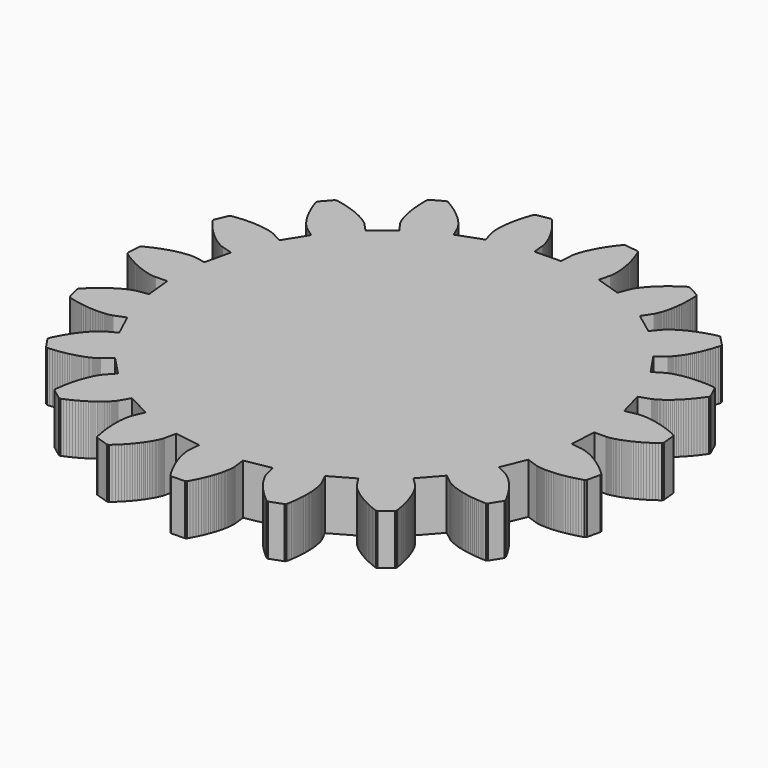
from build123d import *

# Parameters (mm, degrees)
F1_DEPTH = 508


with BuildPart() as f1:
    # F0 (on Top) → F1 (new body)
    with BuildSketch(Plane.XY):
        with BuildLine():
            Line((-9603.0138648, 1999.3428136), (-9486.6818648036, 1999.3468635225))
            add(Edge.make_bspline(
                [(-9533.1965952824, 2455.3824713541), (-9502.7047644041, 2308.1482625823), (-9486.6821416258, 2155.6186806864), (-9486.6818648036, 1999.3468635227)],
                knots=[0.8735232997, 0.8735232997, 0.8735232997, 0.8735232997, 0.9999989074, 0.9999989074, 0.9999989074, 0.9999989074], degree=3))
            Line((-9533.1965952824, 2455.3824713541), (-9533.2410808, 2455.3744136))
            Line((-9533.2410808, 2455.3744136), (-9647.5268568, 2431.5878216))
            Line((-9647.5268568, 2431.5878216), (-9717.9295608, 2687.9977736))
            Line((-9717.9295608, 2687.9977736), (-9607.5208408, 2725.9047336))
            Line((-9607.5208408, 2725.9047336), (-9607.3280556629, 2725.9768848691))
            add(Edge.make_bspline(
                [(-9800.0607330857, 3141.9482313531), (-9722.2973138749, 3011.2963945371), (-9657.4647105246, 2872.0509014997), (-9607.3280556629, 2725.9768848691)],
                knots=[0.6621538595, 0.6621538595, 0.6621538595, 0.6621538595, 0.7941402708, 0.7941402708, 0.7941402708, 0.7941402708], degree=3))
            Line((-9800.0607330857, 3141.948231353), (-9900.3808088, 3082.3703656))
            Line((-9900.3808088, 3082.3703656), (-10050.2265848, 3302.0275336))
            Line((-10050.2265848, 3302.0275336), (-9958.3460478147, 3373.5453460278))
            add(Edge.make_bspline(
                [(-10275.4985599985, 3704.4825641402), (-10158.8666959857, 3605.3134449584), (-10052.53881783, 3494.3906648265), (-9958.3460478146, 3373.5453460277)],
                knots=[0.447110935, 0.447110935, 0.447110935, 0.447110935, 0.58072204, 0.58072204, 0.58072204, 0.58072204], degree=3))
            Line((-10275.4985599985, 3704.4825641403), (-10350.8447288, 3615.7886536))
            Line((-10350.8447288, 3615.7886536), (-10563.8918008, 3774.8901896))
            Line((-10563.8918008, 3774.8901896), (-10500.1274417237, 3872.4951179825))
            add(Edge.make_bspline(
                [(-10907.4279384266, 4082.9072241841), (-10763.8303973859, 4026.5922877078), (-10627.4699039277, 3955.86125775), (-10500.1274417236, 3872.4951179825)],
                knots=[0.2331911594, 0.2331911594, 0.2331911594, 0.2331911594, 0.3655714772, 0.3655714772, 0.3655714772, 0.3655714772], degree=3))
            Line((-10907.4279384265, 4082.9072241841), (-10907.5050328, 4082.7259976))
            Line((-10907.5050328, 4082.7259976), (-10950.0998168, 3974.0404136))
            Line((-10950.0998168, 3974.0404136), (-11203.2646648, 4055.3447976))
            Line((-11203.2646648, 4055.3447976), (-11174.6114328, 4168.5089096))
            Line((-11174.6114328, 4168.5089096), (-11174.5829779644, 4168.6355095043))
            add(Edge.make_bspline(
                [(-11628.2284163068, 4234.5655073528), (-11472.3594729731, 4228.0069192206), (-11320.6144935689, 4205.5004199811), (-11174.5829779643, 4168.6355095043)],
                knots=[0.0259447865, 0.0259447865, 0.0259447865, 0.0259447865, 0.1533998045, 0.1533998045, 0.1533998045, 0.1533998045], degree=3))
            Line((-11628.2284163068, 4234.5655073528), (-11633.2094488, 4118.3022536))
            Line((-11633.2094488, 4118.3022536), (-11899.0560088, 4112.9987336))
            Line((-11899.0560088, 4112.9987336), (-11908.6766526644, 4229.0545916959))
            add(Edge.make_bspline(
                [(-12359.340373963, 4145.0503669471), (-12214.6868569178, 4187.8215900356), (-12063.9252294775, 4216.3633852926), (-11908.6766526644, 4229.0545916959)],
                knots=[0.8213531006, 0.8213531006, 0.8213531006, 0.8213531006, 0.9496488174, 0.9496488174, 0.9496488174, 0.9496488174], degree=3))
            Line((-12359.3403739629, 4145.0503669471), (-12359.2938488, 4144.8747176))
            Line((-12359.2938488, 4144.8747176), (-12326.1498968, 4032.9419976))
            Line((-12326.1498968, 4032.9419976), (-12575.8705048, 3941.6056296))
            Line((-12575.8705048, 3941.6056296), (-12622.7650008, 4048.5071176))
            Line((-12622.7650008, 4048.5071176), (-12622.8338758231, 4048.6532524315))
            add(Edge.make_bspline(
                [(-13021.3866404912, 3822.131690876), (-12897.348558889, 3910.5815329637), (-12763.8997618086, 3986.6865956732), (-12622.8338758231, 4048.6532524315)],
                knots=[0.6085312968, 0.6085312968, 0.6085312968, 0.6085312968, 0.7412241247, 0.7412241247, 0.7412241247, 0.7412241247], degree=3))
            Line((-13021.3866404912, 3822.131690876), (-12953.8265688, 3727.2113416))
            Line((-12953.8265688, 3727.2113416), (-13160.3610808, 3559.7399976))
            Line((-13160.3610808, 3559.7399976), (-13239.1606714034, 3645.3340530318))
            add(Edge.make_bspline(
                [(-13542.94122522, 3302.0745271366), (-13453.5543319971, 3426.6656967517), (-13351.6843139697, 3541.6953721387), (-13239.1606714033, 3645.3340530319)],
                knots=[0.3933460133, 0.3933460133, 0.3933460133, 0.3933460133, 0.5269176555, 0.5269176555, 0.5269176555, 0.5269176555], degree=3))
            Line((-13542.9412252201, 3302.0745271365), (-13448.2263928, 3234.2379816))
            Line((-13448.2263928, 3234.2379816), (-13589.1902968, 3008.7794536))
            Line((-13589.1902968, 3008.7794536), (-13691.8570968, 3064.3363656))
            Line((-13691.8570968, 3064.3363656), (-13691.8798776402, 3064.3478744236))
            add(Edge.make_bspline(
                [(-13867.7762809322, 2640.9763167998), (-13823.499671741, 2789.1300875876), (-13764.2848511316, 2930.8366263076), (-13691.8798776402, 3064.3478744236)],
                knots=[0.1804830407, 0.1804830407, 0.1804830407, 0.1804830407, 0.3120425052, 0.3120425052, 0.3120425052, 0.3120425052], degree=3))
            Line((-13867.7762809322, 2640.9763167999), (-13867.6007128, 2640.9183656))
            Line((-13867.6007128, 2640.9183656), (-13755.7675608, 2607.4452296))
            Line((-13755.7675608, 2607.4452296), (-13815.8883448, 2348.4322856))
            Line((-13815.8883448, 2348.4322856), (-13930.9769832777, 2367.6316661617))
            add(Edge.make_bspline(
                [(-13961.1458648, 1999.3428136), (-13961.1458648, 2124.7848587258), (-13950.8217925222, 2247.8155880167), (-13930.9769832777, 2367.6316661616)],
                knots=[0, 0, 0, 0, 0.1015240791, 0.1015240791, 0.1015240791, 0.1015240791], degree=3))
            add(Edge.make_bspline(
                [(-13959.3991839781, 1910.118183482), (-13960.5600181393, 1939.7156556206), (-13961.1458648, 1969.4608187134), (-13961.1458648, 1999.3428136)],
                knots=[0.9758155887, 0.9758155887, 0.9758155887, 0.9758155887, 1, 1, 1, 1], degree=3))
            Line((-13959.3991839781, 1910.118183482), (-13843.1273048, 1914.7547176))
            Line((-13843.1273048, 1914.7547176), (-13815.8883448, 1650.2533416))
            Line((-13815.8883448, 1650.2533416), (-13930.9756192447, 1631.0457255753))
            add(Edge.make_bspline(
                [(-13809.8342885528, 1188.890350209), (-13864.6606213109, 1329.9002581549), (-13905.6008392703, 1477.8451576725), (-13930.9756192447, 1631.0457255752)],
                knots=[0.7686615868, 0.7686615868, 0.7686615868, 0.7686615868, 0.8984735948, 0.8984735948, 0.8984735948, 0.8984735948], degree=3))
            Line((-13809.8342885528, 1188.890350209), (-13809.6480728, 1188.9568296))
            Line((-13809.6480728, 1188.9568296), (-13700.8365048, 1231.2305576))
            Line((-13700.8365048, 1231.2305576), (-13589.1902968, 989.9061736))
            Line((-13589.1902968, 989.9061736), (-13691.8530328, 934.3431656))
            Line((-13691.8530328, 934.3431656), (-13691.8757045083, 934.3300577601))
            add(Edge.make_bspline(
                [(-13433.2336402329, 555.8579340176), (-13531.7567292961, 672.4070283903), (-13618.5753106051, 799.1689628549), (-13691.8757045083, 934.3300577601)],
                knots=[0.5547694608, 0.5547694608, 0.5547694608, 0.5547694608, 0.6879549673, 0.6879549673, 0.6879549673, 0.6879549673], degree=3))
            Line((-13433.2336402329, 555.8579340176), (-13344.3160088, 630.9432136))
            Line((-13344.3160088, 630.9432136), (-13160.3610808, 438.9456296))
            Line((-13160.3610808, 438.9456296), (-13239.1553657435, 353.3466874634))
            add(Edge.make_bspline(
                [(-12872.068993286, 78.80371775), (-13003.8375703539, 157.7485052172), (-13126.8066823027, 249.8698162513), (-13239.1553657435, 353.3466874634)],
                knots=[0.3397166858, 0.3397166858, 0.3397166858, 0.3397166858, 0.4730802451, 0.4730802451, 0.4730802451, 0.4730802451], degree=3))
            Line((-12872.068993286, 78.80371775), (-12812.1982008, 178.9431016))
            Line((-12812.1982008, 178.9431016), (-12575.8705048, 57.0799976))
            Line((-12575.8705048, 57.0799976), (-12622.7589048, -49.8255544))
            Line((-12622.7589048, -49.8255544), (-12622.8190523596, -49.9741367378))
            add(Edge.make_bspline(
                [(-12186.2871887193, -190.0531618101), (-12338.0259880061, -158.1679267807), (-12484.1050700739, -110.9064575688), (-12622.8190523596, -49.9741367378)],
                knots=[0.128291198, 0.128291198, 0.128291198, 0.128291198, 0.2587712274, 0.2587712274, 0.2587712274, 0.2587712274], degree=3))
            Line((-12186.2871887192, -190.0531618101), (-12186.2751448, -190.0030744))
            Line((-12186.2751448, -190.0030744), (-12162.1492088, -75.7884184))
            Line((-12162.1492088, -75.7884184), (-11899.0560088, -114.3131064))
            Line((-11899.0560088, -114.3131064), (-11908.6684320047, -230.3696365004))
            add(Edge.make_bspline(
                [(-11723.9138648, -237.8891864), (-11786.1244390079, -237.8891864), (-11847.741956448, -235.3500080616), (-11908.6684320048, -230.3696365004)],
                knots=[0, 0, 0, 0, 0.0503489181, 0.0503489181, 0.0503489181, 0.0503489181], degree=3))
            add(Edge.make_bspline(
                [(-11450.3651082082, -221.3331488381), (-11540.0184436995, -232.2627748226), (-11631.3090949535, -237.8891864), (-11723.9138648, -237.8891864)],
                knots=[0.9250521309, 0.9250521309, 0.9250521309, 0.9250521309, 1, 1, 1, 1], degree=3))
            Line((-11450.3651082083, -221.3331488381), (-11464.6123768, -105.6466264))
            Line((-11464.6123768, -105.6466264), (-11203.2646648, -56.6591704))
            Line((-11203.2646648, -56.6591704), (-11174.6033048, -169.8212504))
            Line((-11174.6033048, -169.8212504), (-11174.5678825961, -169.9460714994))
            add(Edge.make_bspline(
                [(-10744.0146845691, -12.4408530361), (-10880.3419816506, -78.9673075028), (-11024.4354544583, -132.0447871225), (-11174.5678825962, -169.9460714994)],
                knots=[0.7155611922, 0.7155611922, 0.7155611922, 0.7155611922, 0.8465958038, 0.8465958038, 0.8465958038, 0.8465958038], degree=3))
            Line((-10744.014684569, -12.4408530361), (-10744.0570488, -12.3473464))
            Line((-10744.0570488, -12.3473464), (-10795.1720088, 92.6034216))
            Line((-10795.1720088, 92.6034216), (-10563.8918008, 223.7954376))
            Line((-10563.8918008, 223.7954376), (-10500.1203912836, 126.1951248844))
            add(Edge.make_bspline(
                [(-10144.2391736468, 415.0969642894), (-10252.4797214366, 307.1667853065), (-10371.7154439888, 210.2575221649), (-10500.1203912836, 126.1951248844)],
                knots=[0.5009408945, 0.5009408945, 0.5009408945, 0.5009408945, 0.6344260797, 0.6344260797, 0.6344260797, 0.6344260797], degree=3))
            Line((-10144.2391736467, 415.0969642894), (-10226.3766008, 497.4773896))
            Line((-10226.3766008, 497.4773896), (-10050.2265848, 696.6580936))
            Line((-10050.2265848, 696.6580936), (-9958.3408022633, 625.1470110179))
            add(Edge.make_bspline(
                [(-9714.9765376319, 1013.6322864737), (-9782.8750578042, 875.5125512748), (-9864.5981533991, 745.4157854051), (-9958.3408022633, 625.1470110179)],
                knots=[0.2863022292, 0.2863022292, 0.2863022292, 0.2863022292, 0.4192754798, 0.4192754798, 0.4192754798, 0.4192754798], degree=3))
            Line((-9714.9765376318, 1013.6322864738), (-9715.0644408, 1013.6785416))
            Line((-9715.0644408, 1013.6785416), (-9819.8628088, 1065.1023656))
            Line((-9819.8628088, 1065.1023656), (-9717.9295608, 1310.6878536))
            Line((-9717.9295608, 1310.6878536), (-9607.5188088, 1272.7869896))
            Line((-9607.5188088, 1272.7869896), (-9607.3223231002, 1272.7254444684))
            add(Edge.make_bspline(
                [(-9504.0296804573, 1719.3764080671), (-9523.2947505668, 1565.0595823636), (-9558.2764720705, 1415.6250872078), (-9607.3223231002, 1272.7254444682)],
                knots=[0.0767369798, 0.0767369798, 0.0767369798, 0.0767369798, 0.2058546987, 0.2058546987, 0.2058546987, 0.2058546987], degree=3))
            Line((-9504.0296804573, 1719.3764080671), (-9619.6823608, 1733.9656456))
            Line((-9619.6823608, 1733.9656456), (-9603.0138648, 1999.3428136))
        make_face()
        Polygon((-10769.6866648, 490.1764136), (-10744.4898648, 506.2292136), (-10737.1746648, 438.5636136), (-10731.6882648, 370.0852136), (-10790.0066648, 406.2548136), (-10846.9026648, 444.0500136), (-10820.8930648, 458.8836136), (-10795.0866648, 474.3268136), align=None, mode=Mode.SUBTRACT)
        Polygon((-10604.0786648, 569.6276136), (-10580.2128472481, 588.6393665651), (-10522.5954648, 517.6084136), (-10547.5890648, 497.6948136), (-10572.9890648, 478.1876136), (-10598.5922648, 459.0868136), (-10642.2802648, 465.3860136), (-10659.7554648, 490.1764136), (-10652.6434648, 532.8484136), (-10628.0562648, 551.1364136), align=None, mode=Mode.SUBTRACT)
        Polygon((-10335.0418648, 691.7508136), (-10423.7755314892, 775.3365729088), (-10403.5202648, 797.4148136), (-10383.4034648, 819.7668136), (-10363.8962648, 842.3220136), (-10352.9234648, 792.7412136), (-10343.3730648, 742.5508136), align=None, mode=Mode.SUBTRACT)
        Polygon((-9833.5442648, 1743.9204136), (-9954.4565245396, 1760.322188744), (-9954.4482648, 1760.3796136), (-9950.5874648, 1790.0468136), (-9947.3362648, 1819.9172136), (-9944.4914648, 1849.5844136), (-9906.8994648, 1815.6500136), (-9869.9170648, 1780.4964136), align=None, mode=Mode.SUBTRACT)
        Polygon((-10005.2482648, 2143.8180136), (-10007.8898648, 2172.6724136), (-9826.0258648, 2191.1636136), (-9823.1810648, 2159.2612136), (-9820.7426648, 2127.3588136), (-9849.1906648, 2093.8308136), (-9970.9074648, 2087.7348136), (-10003.2162648, 2114.9636136), align=None, mode=Mode.SUBTRACT)
        Polygon((-10357.1906648, 3286.0052136), (-10401.7274454983, 3244.1840902613), (-10422.6210648, 3266.2948136), (-10444.1602648, 3287.8340136), (-10465.9026648, 3309.1700136), (-10467.3250648, 3352.4516136), (-10446.5986648, 3374.8036136), (-10402.5042648, 3375.2100136), (-10379.7458648, 3352.8580136), (-10357.1906648, 3330.0996136), align=None, mode=Mode.SUBTRACT)
        Polygon((-11313.1286691555, 3768.4729399437), (-11313.150399452, 3768.3789362906), (-11313.1730613718, 3768.2809025044), (-11313.2466648, 3768.4020136), align=None, mode=Mode.SUBTRACT)
        with BuildLine():
            add(Edge.make_bspline(
                [(-13542.94122522, 3302.0745271366), (-13453.5543319971, 3426.6656967517), (-13351.6843139697, 3541.6953721387), (-13239.1606714033, 3645.3340530319)],
                knots=[0.3933460133, 0.3933460133, 0.3933460133, 0.3933460133, 0.5269176555, 0.5269176555, 0.5269176555, 0.5269176555], degree=3))
            Line((-13239.1606714034, 3645.3340530318), (-13239.4262008, 3645.6224776))
            Line((-13239.4262008, 3645.6224776), (-13240.1902328, 3646.4068296))
            Line((-13240.1902328, 3646.4068296), (-13241.5029048, 3647.7093416))
            Line((-13241.5029048, 3647.7093416), (-13243.3865688, 3649.5096936))
            Line((-13243.3865688, 3649.5096936), (-13245.8574808, 3651.7875656))
            Line((-13245.8574808, 3651.7875656), (-13248.9339288, 3654.5206056))
            Line((-13248.9339288, 3654.5206056), (-13252.6342008, 3657.6884936))
            Line((-13252.6342008, 3657.6884936), (-13256.9745528, 3661.2668456))
            Line((-13256.9745528, 3661.2668456), (-13261.9712408, 3665.2353416))
            Line((-13261.9712408, 3665.2353416), (-13267.6384888, 3669.5716296))
            Line((-13267.6384888, 3669.5716296), (-13273.9945848, 3674.2492936))
            Line((-13273.9945848, 3674.2492936), (-13281.0496888, 3679.2480136))
            Line((-13281.0496888, 3679.2480136), (-13288.8200568, 3684.5393416))
            Line((-13288.8200568, 3684.5393416), (-13297.3178808, 3690.1009256))
            Line((-13297.3178808, 3690.1009256), (-13306.5573848, 3695.9083816))
            Line((-13306.5573848, 3695.9083816), (-13316.5466968, 3701.9332616))
            Line((-13316.5466968, 3701.9332616), (-13327.3000408, 3708.1532136))
            Line((-13327.3000408, 3708.1532136), (-13338.8255448, 3714.5418216))
            Line((-13338.8255448, 3714.5418216), (-13351.1333688, 3721.0706376))
            Line((-13351.1333688, 3721.0706376), (-13364.2316408, 3727.7132456))
            Line((-13364.2316408, 3727.7132456), (-13378.1305208, 3734.4432296))
            Line((-13378.1305208, 3734.4432296), (-13392.8361048, 3741.2341736))
            Line((-13392.8361048, 3741.2341736), (-13393.4723435948, 3741.5138454128))
            add(Edge.make_bspline(
                [(-13657.2145353256, 3443.5092487252), (-13577.5480837532, 3549.9866386154), (-13489.2914904386, 3649.6640335823), (-13393.4723435948, 3741.5138454129)],
                knots=[0.4063946667, 0.4063946667, 0.4063946667, 0.4063946667, 0.5138581844, 0.5138581844, 0.5138581844, 0.5138581844], degree=3))
            Line((-13657.2145353255, 3443.5092487252), (-13656.7807128, 3442.7801096))
            Line((-13656.7807128, 3442.7801096), (-13648.2422488, 3429.0153416))
            Line((-13648.2422488, 3429.0153416), (-13639.8643128, 3416.0430536))
            Line((-13639.8643128, 3416.0430536), (-13631.6692568, 3403.8551176))
            Line((-13631.6692568, 3403.8551176), (-13623.6855288, 3392.4373096))
            Line((-13623.6855288, 3392.4373096), (-13615.9354808, 3381.7794696))
            Line((-13615.9354808, 3381.7794696), (-13608.4475608, 3371.8673736))
            Line((-13608.4475608, 3371.8673736), (-13601.2461528, 3362.6888296))
            Line((-13601.2461528, 3362.6888296), (-13594.3536088, 3354.2296136))
            Line((-13594.3536088, 3354.2296136), (-13587.7943128, 3346.4755016))
            Line((-13587.7943128, 3346.4755016), (-13581.5926488, 3339.4102376))
            Line((-13581.5926488, 3339.4102376), (-13575.7689368, 3333.0195976))
            Line((-13575.7689368, 3333.0195976), (-13570.3495928, 3327.2832616))
            Line((-13570.3495928, 3327.2832616), (-13565.3529048, 3322.1890376))
            Line((-13565.3529048, 3322.1890376), (-13560.8032568, 3317.7145736))
            Line((-13560.8032568, 3317.7145736), (-13556.7189368, 3313.8456456))
            Line((-13556.7189368, 3313.8456456), (-13553.1243288, 3310.5599016))
            Line((-13553.1243288, 3310.5599016), (-13550.0356888, 3307.8410856))
            Line((-13550.0356888, 3307.8410856), (-13547.4733368, 3305.6668456))
            Line((-13547.4733368, 3305.6668456), (-13545.4555608, 3304.0168616))
            Line((-13545.4555608, 3304.0168616), (-13544.0026808, 3302.8728456))
            Line((-13544.0026808, 3302.8728456), (-13543.1309528, 3302.2104136))
            Line((-13543.1309528, 3302.2104136), (-13542.9412252201, 3302.0745271365))
        make_face()
        with BuildLine():
            add(Edge.make_bspline(
                [(-13657.2145353256, 3443.5092487252), (-13577.5480837532, 3549.9866386154), (-13489.2914904386, 3649.6640335823), (-13393.4723435948, 3741.5138454129)],
                knots=[0.4063946667, 0.4063946667, 0.4063946667, 0.4063946667, 0.5138581844, 0.5138581844, 0.5138581844, 0.5138581844], degree=3))
            Line((-13393.4723435948, 3741.5138454128), (-13408.3544888, 3748.0555976))
            Line((-13408.3544888, 3748.0555976), (-13424.6938008, 3754.8851496))
            Line((-13424.6938008, 3754.8851496), (-13441.8581048, 3761.6903176))
            Line((-13441.8581048, 3761.6903176), (-13459.8494328, 3768.4426536))
            Line((-13459.8494328, 3768.4426536), (-13478.6738808, 3775.1177736))
            Line((-13478.6738808, 3775.1177736), (-13498.3355128, 3781.6851976))
            Line((-13498.3355128, 3781.6851976), (-13518.8343288, 3788.1164776))
            Line((-13518.8343288, 3788.1164776), (-13540.1703288, 3794.3831656))
            Line((-13540.1703288, 3794.3831656), (-13562.3496088, 3800.4547816))
            Line((-13562.3496088, 3800.4547816), (-13585.3660728, 3806.3049096))
            Line((-13585.3660728, 3806.3049096), (-13609.2217528, 3811.9030696))
            Line((-13609.2217528, 3811.9030696), (-13633.9146168, 3817.2228456))
            Line((-13633.9146168, 3817.2228456), (-13659.4426328, 3822.2317256))
            Line((-13659.4426328, 3822.2317256), (-13675.3918008, 3817.2065896))
            Line((-13675.3918008, 3817.2065896), (-13766.7281688, 3713.9261256))
            Line((-13766.7281688, 3713.9261256), (-13769.7660088, 3697.4831816))
            Line((-13769.7660088, 3697.4831816), (-13761.6725528, 3672.7598376))
            Line((-13761.6725528, 3672.7598376), (-13753.3758968, 3648.9021256))
            Line((-13753.3758968, 3648.9021256), (-13744.9024568, 3625.9100456))
            Line((-13744.9024568, 3625.9100456), (-13736.2827128, 3603.7815656))
            Line((-13736.2827128, 3603.7815656), (-13727.5430808, 3582.5126216))
            Line((-13727.5430808, 3582.5126216), (-13718.7160728, 3562.1011816))
            Line((-13718.7160728, 3562.1011816), (-13709.8281048, 3542.5431816))
            Line((-13709.8281048, 3542.5431816), (-13700.9055928, 3523.8325256))
            Line((-13700.9055928, 3523.8325256), (-13691.9790168, 3505.9651496))
            Line((-13691.9790168, 3505.9651496), (-13683.0768248, 3488.9329256))
            Line((-13683.0768248, 3488.9329256), (-13674.2234008, 3472.7297576))
            Line((-13674.2234008, 3472.7297576), (-13665.4492248, 3457.3495496))
            Line((-13665.4492248, 3457.3495496), (-13657.2145353255, 3443.5092487252))
        make_face()
        with BuildLine():
            add(Edge.make_bspline(
                [(-13083.5615893126, 3993.0951740829), (-12974.4072104198, 4067.6773031445), (-12858.8143137381, 4133.5292146014), (-12737.7883932193, 4189.6454145018)],
                knots=[0.6215801777, 0.6215801777, 0.6215801777, 0.6215801777, 0.7282679144, 0.7282679144, 0.7282679144, 0.7282679144], degree=3))
            Line((-12737.7883932193, 4189.6454145018), (-12749.2813848, 4200.2426536))
            Line((-12749.2813848, 4200.2426536), (-12762.5178328, 4212.0059016))
            Line((-12762.5178328, 4212.0059016), (-12776.5406648, 4224.0150216))
            Line((-12776.5406648, 4224.0150216), (-12791.3661368, 4236.2456296))
            Line((-12791.3661368, 4236.2456296), (-12807.0023768, 4248.6713096))
            Line((-12807.0023768, 4248.6713096), (-12823.4656408, 4261.2676776))
            Line((-12823.4656408, 4261.2676776), (-12840.7660888, 4274.0042536))
            Line((-12840.7660888, 4274.0042536), (-12858.9138808, 4286.8607176))
            Line((-12858.9138808, 4286.8607176), (-12877.9171448, 4299.8045576))
            Line((-12877.9171448, 4299.8045576), (-12897.7880728, 4312.8113896))
            Line((-12897.7880728, 4312.8113896), (-12918.5327608, 4325.8527656))
            Line((-12918.5327608, 4325.8527656), (-12940.1613688, 4338.9002376))
            Line((-12940.1613688, 4338.9002376), (-12962.6799928, 4351.9273896))
            Line((-12962.6799928, 4351.9273896), (-12979.3952248, 4352.3520776))
            Line((-12979.3952248, 4352.3520776), (-13099.3177688, 4284.3268136))
            Line((-13099.3177688, 4284.3268136), (-13107.5311128, 4269.7614376))
            Line((-13107.5311128, 4269.7614376), (-13107.9050008, 4243.7498056))
            Line((-13107.9050008, 4243.7498056), (-13107.8034008, 4218.4900136))
            Line((-13107.8034008, 4218.4900136), (-13107.2547608, 4193.9922216))
            Line((-13107.2547608, 4193.9922216), (-13106.2854968, 4170.2625256))
            Line((-13106.2854968, 4170.2625256), (-13104.9281208, 4147.3090536))
            Line((-13104.9281208, 4147.3090536), (-13103.2049848, 4125.1379016))
            Line((-13103.2049848, 4125.1379016), (-13101.1486008, 4103.7531336))
            Line((-13101.1486008, 4103.7531336), (-13098.7853848, 4083.1588136))
            Line((-13098.7853848, 4083.1588136), (-13096.1458168, 4063.3610376))
            Line((-13096.1458168, 4063.3610376), (-13093.2542808, 4044.3618376))
            Line((-13093.2542808, 4044.3618376), (-13090.1432888, 4026.1632456))
            Line((-13090.1432888, 4026.1632456), (-13086.8372248, 4008.7652616))
            Line((-13086.8372248, 4008.7652616), (-13083.5615893124, 3993.0951740828))
        make_face()
        with BuildLine():
            add(Edge.make_bspline(
                [(-13021.3866404912, 3822.131690876), (-12897.348558889, 3910.5815329637), (-12763.8997618086, 3986.6865956732), (-12622.8338758231, 4048.6532524315)],
                knots=[0.6085312968, 0.6085312968, 0.6085312968, 0.6085312968, 0.7412241247, 0.7412241247, 0.7412241247, 0.7412241247], degree=3))
            Line((-12622.8338758231, 4048.6532524315), (-12623.2323608, 4049.4987336))
            Line((-12623.2323608, 4049.4987336), (-12624.0532888, 4051.1568456))
            Line((-12624.0532888, 4051.1568456), (-12625.2481048, 4053.4712936))
            Line((-12625.2481048, 4053.4712936), (-12626.8472888, 4056.4278536))
            Line((-12626.8472888, 4056.4278536), (-12628.8691288, 4060.0123016))
            Line((-12628.8691288, 4060.0123016), (-12631.3400408, 4064.2083816))
            Line((-12631.3400408, 4064.2083816), (-12634.2823768, 4069.0039016))
            Line((-12634.2823768, 4069.0039016), (-12637.7205208, 4074.3805736))
            Line((-12637.7205208, 4074.3805736), (-12641.6727608, 4080.3201096))
            Line((-12641.6727608, 4080.3201096), (-12646.1655128, 4086.8082856))
            Line((-12646.1655128, 4086.8082856), (-12651.2150328, 4093.8268136))
            Line((-12651.2150328, 4093.8268136), (-12656.8477368, 4101.3553736))
            Line((-12656.8477368, 4101.3553736), (-12663.0778488, 4109.3756776))
            Line((-12663.0778488, 4109.3756776), (-12669.9317848, 4117.8674056))
            Line((-12669.9317848, 4117.8674056), (-12677.4237688, 4126.8102376))
            Line((-12677.4237688, 4126.8102376), (-12685.5741208, 4136.1838536))
            Line((-12685.5741208, 4136.1838536), (-12694.4011288, 4145.9679336))
            Line((-12694.4011288, 4145.9679336), (-12703.9210488, 4156.1380936))
            Line((-12703.9210488, 4156.1380936), (-12714.1542008, 4166.6760456))
            Line((-12714.1542008, 4166.6760456), (-12725.1148088, 4177.5533416))
            Line((-12725.1148088, 4177.5533416), (-12736.8191288, 4188.7516936))
            Line((-12736.8191288, 4188.7516936), (-12737.7883932193, 4189.6454145018))
            add(Edge.make_bspline(
                [(-13083.5615893126, 3993.0951740829), (-12974.4072104198, 4067.6773031445), (-12858.8143137381, 4133.5292146014), (-12737.7883932193, 4189.6454145018)],
                knots=[0.6215801777, 0.6215801777, 0.6215801777, 0.6215801777, 0.7282679144, 0.7282679144, 0.7282679144, 0.7282679144], degree=3))
            Line((-13083.5615893124, 3993.0951740828), (-13083.3686008, 3992.1719496))
            Line((-13083.3686008, 3992.1719496), (-13079.7638328, 3976.3812776))
            Line((-13079.7638328, 3976.3812776), (-13076.0493368, 3961.3912136))
            Line((-13076.0493368, 3961.3912136), (-13072.2576248, 3947.2017576))
            Line((-13072.2576248, 3947.2017576), (-13068.4130808, 3933.8108776))
            Line((-13068.4130808, 3933.8108776), (-13064.5441528, 3921.2145096))
            Line((-13064.5441528, 3921.2145096), (-13060.6813208, 3909.4085896))
            Line((-13060.6813208, 3909.4085896), (-13056.8489688, 3898.3890536))
            Line((-13056.8489688, 3898.3890536), (-13053.0755448, 3888.1498056))
            Line((-13053.0755448, 3888.1498056), (-13049.3915288, 3878.6847496))
            Line((-13049.3915288, 3878.6847496), (-13045.8192728, 3869.9898216))
            Line((-13045.8192728, 3869.9898216), (-13042.3872248, 3862.0528296))
            Line((-13042.3872248, 3862.0528296), (-13039.1218008, 3854.8697096))
            Line((-13039.1218008, 3854.8697096), (-13036.0514488, 3848.4262376))
            Line((-13036.0514488, 3848.4262376), (-13033.2005528, 3842.7183496))
            Line((-13033.2005528, 3842.7183496), (-13030.5955288, 3837.7318216))
            Line((-13030.5955288, 3837.7318216), (-13028.2607608, 3833.4585256))
            Line((-13028.2607608, 3833.4585256), (-13026.2226648, 3829.8822056))
            Line((-13026.2226648, 3829.8822056), (-13024.5056248, 3826.9947336))
            Line((-13024.5056248, 3826.9947336), (-13023.1319928, 3824.7798536))
            Line((-13023.1319928, 3824.7798536), (-13022.1302168, 3823.2253736))
            Line((-13022.1302168, 3823.2253736), (-13021.5185848, 3822.3170696))
            Line((-13021.5185848, 3822.3170696), (-13021.3866404912, 3822.131690876))
        make_face()
        with BuildLine():
            add(Edge.make_bspline(
                [(-12362.4708094618, 4326.9477052126), (-12235.978628718, 4361.570142365), (-12105.3395480861, 4386.1572385811), (-11971.4625859846, 4399.7999754423)],
                knots=[0.8341257104, 0.8341257104, 0.8341257104, 0.8341257104, 0.9372859262, 0.9372859262, 0.9372859262, 0.9372859262], degree=3))
            Line((-11971.4625859845, 4399.7999754424), (-11979.0924248, 4413.9298056))
            Line((-11979.0924248, 4413.9298056), (-11987.7914168, 4429.3526856))
            Line((-11987.7914168, 4429.3526856), (-11997.1569048, 4445.2652776))
            Line((-11997.1569048, 4445.2652776), (-12007.2071768, 4461.6452296))
            Line((-12007.2071768, 4461.6452296), (-12017.9625528, 4478.4762856))
            Line((-12017.9625528, 4478.4762856), (-12029.4433528, 4495.7340616))
            Line((-12029.4433528, 4495.7340616), (-12041.6698968, 4513.3982376))
            Line((-12041.6698968, 4513.3982376), (-12054.6604728, 4531.4505256))
            Line((-12054.6604728, 4531.4505256), (-12068.4313368, 4549.8624776))
            Line((-12068.4313368, 4549.8624776), (-12083.0028088, 4568.6178376))
            Line((-12083.0028088, 4568.6178376), (-12098.3891128, 4587.6881576))
            Line((-12098.3891128, 4587.6881576), (-12114.6085368, 4607.0531176))
            Line((-12114.6085368, 4607.0531176), (-12131.6753048, 4626.6842696))
            Line((-12131.6753048, 4626.6842696), (-12147.3481208, 4632.5140776))
            Line((-12147.3481208, 4632.5140776), (-12282.8622008, 4607.1140776))
            Line((-12282.8622008, 4607.1140776), (-12295.3590008, 4596.0031016))
            Line((-12295.3590008, 4596.0031016), (-12304.1575608, 4571.5215656))
            Line((-12304.1575608, 4571.5215656), (-12312.2632088, 4547.5988296))
            Line((-12312.2632088, 4547.5988296), (-12319.7003288, 4524.2491176))
            Line((-12319.7003288, 4524.2491176), (-12326.4892408, 4501.4927496))
            Line((-12326.4892408, 4501.4927496), (-12332.6563608, 4479.3398856))
            Line((-12332.6563608, 4479.3398856), (-12338.2281048, 4457.8108456))
            Line((-12338.2281048, 4457.8108456), (-12343.2247928, 4436.9178216))
            Line((-12343.2247928, 4436.9178216), (-12347.6769048, 4416.6730056))
            Line((-12347.6769048, 4416.6730056), (-12351.6088248, 4397.0885896))
            Line((-12351.6088248, 4397.0885896), (-12355.0429048, 4378.1808296))
            Line((-12355.0429048, 4378.1808296), (-12358.0096248, 4359.9578536))
            Line((-12358.0096248, 4359.9578536), (-12360.5313368, 4342.4298216))
            Line((-12360.5313368, 4342.4298216), (-12362.4708094617, 4326.9477052125))
        make_face()
        with BuildLine():
            add(Edge.make_bspline(
                [(-12359.340373963, 4145.0503669471), (-12214.6868569178, 4187.8215900356), (-12063.9252294775, 4216.3633852926), (-11908.6766526644, 4229.0545916959)],
                knots=[0.8213531006, 0.8213531006, 0.8213531006, 0.8213531006, 0.9496488174, 0.9496488174, 0.9496488174, 0.9496488174], degree=3))
            Line((-11908.6766526644, 4229.0545916959), (-11908.6998808, 4229.3347976))
            Line((-11908.6998808, 4229.3347976), (-11908.8218008, 4230.4239496))
            Line((-11908.8218008, 4230.4239496), (-11909.0575128, 4232.2588456))
            Line((-11909.0575128, 4232.2588456), (-11909.4374968, 4234.8354216))
            Line((-11909.4374968, 4234.8354216), (-11909.9881688, 4238.1496136))
            Line((-11909.9881688, 4238.1496136), (-11910.7379768, 4242.1973576))
            Line((-11910.7379768, 4242.1973576), (-11911.7133368, 4246.9684936))
            Line((-11911.7133368, 4246.9684936), (-11912.9386328, 4252.4589576))
            Line((-11912.9386328, 4252.4589576), (-11914.4443448, 4258.6606216))
            Line((-11914.4443448, 4258.6606216), (-11916.2548568, 4265.5633256))
            Line((-11916.2548568, 4265.5633256), (-11918.3945528, 4273.1589416))
            Line((-11918.3945528, 4273.1589416), (-11920.8939128, 4281.4352776))
            Line((-11920.8939128, 4281.4352776), (-11923.7752888, 4290.3842056))
            Line((-11923.7752888, 4290.3842056), (-11927.0650968, 4299.9935336))
            Line((-11927.0650968, 4299.9935336), (-11930.7897528, 4310.2510696))
            Line((-11930.7897528, 4310.2510696), (-11934.9716088, 4321.1425896))
            Line((-11934.9716088, 4321.1425896), (-11939.6370808, 4332.6538696))
            Line((-11939.6370808, 4332.6538696), (-11944.8085208, 4344.7747496))
            Line((-11944.8085208, 4344.7747496), (-11950.5123448, 4357.4849096))
            Line((-11950.5123448, 4357.4849096), (-11956.7688728, 4370.7741896))
            Line((-11956.7688728, 4370.7741896), (-11963.6024888, 4384.6222696))
            Line((-11963.6024888, 4384.6222696), (-11971.0375768, 4399.0128936))
            Line((-11971.0375768, 4399.0128936), (-11971.4625859845, 4399.7999754424))
            add(Edge.make_bspline(
                [(-12362.4708094618, 4326.9477052126), (-12235.978628718, 4361.570142365), (-12105.3395480861, 4386.1572385811), (-11971.4625859846, 4399.7999754423)],
                knots=[0.8341257104, 0.8341257104, 0.8341257104, 0.8341257104, 0.9372859262, 0.9372859262, 0.9372859262, 0.9372859262], degree=3))
            Line((-12362.4708094617, 4326.9477052125), (-12362.6385208, 4325.6089256))
            Line((-12362.6385208, 4325.6089256), (-12364.3575928, 4309.5032936))
            Line((-12364.3575928, 4309.5032936), (-12365.7109048, 4294.1190216))
            Line((-12365.7109048, 4294.1190216), (-12366.7309688, 4279.4683016))
            Line((-12366.7309688, 4279.4683016), (-12367.4442008, 4265.5531656))
            Line((-12367.4442008, 4265.5531656), (-12367.8749848, 4252.3837736))
            Line((-12367.8749848, 4252.3837736), (-12368.0538008, 4239.9621576))
            Line((-12368.0538008, 4239.9621576), (-12368.0070648, 4228.2964456))
            Line((-12368.0070648, 4228.2964456), (-12367.7632248, 4217.3866376))
            Line((-12367.7632248, 4217.3866376), (-12367.3507288, 4207.2388296))
            Line((-12367.3507288, 4207.2388296), (-12366.7959928, 4197.8550536))
            Line((-12366.7959928, 4197.8550536), (-12366.1274648, 4189.2332776))
            Line((-12366.1274648, 4189.2332776), (-12365.3715608, 4181.3795976))
            Line((-12365.3715608, 4181.3795976), (-12364.5607928, 4174.2899496))
            Line((-12364.5607928, 4174.2899496), (-12363.7175128, 4167.9643336))
            Line((-12363.7175128, 4167.9643336), (-12362.8722008, 4162.4027496))
            Line((-12362.8722008, 4162.4027496), (-12362.0512728, 4157.6011336))
            Line((-12362.0512728, 4157.6011336), (-12361.2852088, 4153.5574536))
            Line((-12361.2852088, 4153.5574536), (-12360.5983928, 4150.2676456))
            Line((-12360.5983928, 4150.2676456), (-12360.0192728, 4147.7276456))
            Line((-12360.0192728, 4147.7276456), (-12359.5742648, 4145.9333896))
            Line((-12359.5742648, 4145.9333896), (-12359.3403739629, 4145.0503669471))
        make_face()
        with BuildLine():
            add(Edge.make_bspline(
                [(-11572.3516271237, 4407.6601880813), (-11437.8484979552, 4399.3241742164), (-11306.3288751578, 4379.9693704926), (-11178.6845316744, 4350.4875498524)],
                knots=[0.038197413, 0.038197413, 0.038197413, 0.038197413, 0.1407010901, 0.1407010901, 0.1407010901, 0.1407010901], degree=3))
            Line((-11178.6845316745, 4350.4875498524), (-11181.2520088, 4365.9563176))
            Line((-11181.2520088, 4365.9563176), (-11184.4727288, 4383.3685256))
            Line((-11184.4727288, 4383.3685256), (-11188.1628408, 4401.4594216))
            Line((-11188.1628408, 4401.4594216), (-11192.3487608, 4420.2168136))
            Line((-11192.3487608, 4420.2168136), (-11197.0569048, 4439.6264776))
            Line((-11197.0569048, 4439.6264776), (-11202.3136888, 4459.6782536))
            Line((-11202.3136888, 4459.6782536), (-11208.1414648, 4480.3558856))
            Line((-11208.1414648, 4480.3558856), (-11214.5646168, 4501.6471816))
            Line((-11214.5646168, 4501.6471816), (-11221.6115928, 4523.5338536))
            Line((-11221.6115928, 4523.5338536), (-11229.3027128, 4546.0037096))
            Line((-11229.3027128, 4546.0037096), (-11237.6643928, 4569.0364296))
            Line((-11237.6643928, 4569.0364296), (-11246.7169528, 4592.6177896))
            Line((-11246.7169528, 4592.6177896), (-11256.4868088, 4616.7274696))
            Line((-11256.4868088, 4616.7274696), (-11269.4164248, 4627.3304456))
            Line((-11269.4164248, 4627.3304456), (-11405.8347448, 4647.3070376))
            Line((-11405.8347448, 4647.3070376), (-11421.2616888, 4640.8574696))
            Line((-11421.2616888, 4640.8574696), (-11437.5339448, 4620.5598216))
            Line((-11437.5339448, 4620.5598216), (-11452.9690168, 4600.5649416))
            Line((-11452.9690168, 4600.5649416), (-11467.5811288, 4580.8951816))
            Line((-11467.5811288, 4580.8951816), (-11481.3926328, 4561.5749256))
            Line((-11481.3926328, 4561.5749256), (-11494.4197848, 4542.6265256))
            Line((-11494.4197848, 4542.6265256), (-11506.6788408, 4524.0723336))
            Line((-11506.6788408, 4524.0723336), (-11518.1901208, 4505.9326696))
            Line((-11518.1901208, 4505.9326696), (-11528.9739448, 4488.2298856))
            Line((-11528.9739448, 4488.2298856), (-11539.0506328, 4470.9843016))
            Line((-11539.0506328, 4470.9843016), (-11548.4384728, 4454.2162376))
            Line((-11548.4384728, 4454.2162376), (-11557.1618488, 4437.9439816))
            Line((-11557.1618488, 4437.9439816), (-11565.2390488, 4422.1858216))
            Line((-11565.2390488, 4422.1858216), (-11572.3516271238, 4407.6601880813))
        make_face()
        with BuildLine():
            add(Edge.make_bspline(
                [(-11628.2284163068, 4234.5655073528), (-11472.3594729731, 4228.0069192206), (-11320.6144935689, 4205.5004199811), (-11174.5829779643, 4168.6355095043)],
                knots=[0.0259447865, 0.0259447865, 0.0259447865, 0.0259447865, 0.1533998045, 0.1533998045, 0.1533998045, 0.1533998045], degree=3))
            Line((-11174.5829779644, 4168.6355095043), (-11174.3716568, 4169.5757096))
            Line((-11174.3716568, 4169.5757096), (-11173.9998008, 4171.3882536))
            Line((-11173.9998008, 4171.3882536), (-11173.5222808, 4173.9506056))
            Line((-11173.5222808, 4173.9506056), (-11172.9675448, 4177.2647976))
            Line((-11172.9675448, 4177.2647976), (-11172.3620088, 4181.3348936))
            Line((-11172.3620088, 4181.3348936), (-11171.7341208, 4186.1649576))
            Line((-11171.7341208, 4186.1649576), (-11171.1102968, 4191.7570216))
            Line((-11171.1102968, 4191.7570216), (-11170.5210168, 4198.1090536))
            Line((-11170.5210168, 4198.1090536), (-11169.9926968, 4205.2251176))
            Line((-11169.9926968, 4205.2251176), (-11169.5517528, 4213.1052136))
            Line((-11169.5517528, 4213.1052136), (-11169.2266328, 4221.7452776))
            Line((-11169.2266328, 4221.7452776), (-11169.0457848, 4231.1453096))
            Line((-11169.0457848, 4231.1453096), (-11169.0376568, 4241.3012456))
            Line((-11169.0376568, 4241.3012456), (-11169.2306968, 4252.2110536))
            Line((-11169.2306968, 4252.2110536), (-11169.6492888, 4263.8706696))
            Line((-11169.6492888, 4263.8706696), (-11170.3239128, 4276.2739976))
            Line((-11170.3239128, 4276.2739976), (-11171.2789528, 4289.4169736))
            Line((-11171.2789528, 4289.4169736), (-11172.5469208, 4303.2914696))
            Line((-11172.5469208, 4303.2914696), (-11174.1501688, 4317.8913896))
            Line((-11174.1501688, 4317.8913896), (-11176.1171448, 4333.2065736))
            Line((-11176.1171448, 4333.2065736), (-11178.4762968, 4349.2329576))
            Line((-11178.4762968, 4349.2329576), (-11178.6845316745, 4350.4875498524))
            add(Edge.make_bspline(
                [(-11572.3516271237, 4407.6601880813), (-11437.8484979552, 4399.3241742164), (-11306.3288751578, 4379.9693704926), (-11178.6845316744, 4350.4875498524)],
                knots=[0.038197413, 0.038197413, 0.038197413, 0.038197413, 0.1407010901, 0.1407010901, 0.1407010901, 0.1407010901], degree=3))
            Line((-11572.3516271238, 4407.6601880813), (-11572.6944568, 4406.9600456))
            Line((-11572.6944568, 4406.9600456), (-11579.5483928, 4392.2829096))
            Line((-11579.5483928, 4392.2829096), (-11585.8252408, 4378.1747336))
            Line((-11585.8252408, 4378.1747336), (-11591.5473528, 4364.6477096))
            Line((-11591.5473528, 4364.6477096), (-11596.7370808, 4351.7180936))
            Line((-11596.7370808, 4351.7180936), (-11601.4228728, 4339.4021416))
            Line((-11601.4228728, 4339.4021416), (-11605.6250488, 4327.7120456))
            Line((-11605.6250488, 4327.7120456), (-11609.3700248, 4316.6620296))
            Line((-11609.3700248, 4316.6620296), (-11612.6801528, 4306.2663176))
            Line((-11612.6801528, 4306.2663176), (-11615.5859128, 4296.5330376))
            Line((-11615.5859128, 4296.5330376), (-11618.1076248, 4287.4764136))
            Line((-11618.1076248, 4287.4764136), (-11620.2737368, 4279.1066056))
            Line((-11620.2737368, 4279.1066056), (-11622.1106648, 4271.4317416))
            Line((-11622.1106648, 4271.4317416), (-11623.6448248, 4264.4619816))
            Line((-11623.6448248, 4264.4619816), (-11624.9006008, 4258.2054536))
            Line((-11624.9006008, 4258.2054536), (-11625.9064408, 4252.6702856))
            Line((-11625.9064408, 4252.6702856), (-11626.6907928, 4247.8646056))
            Line((-11626.6907928, 4247.8646056), (-11627.2780408, 4243.7904456))
            Line((-11627.2780408, 4243.7904456), (-11627.6966328, 4240.4559336))
            Line((-11627.6966328, 4240.4559336), (-11627.9729848, 4237.8651336))
            Line((-11627.9729848, 4237.8651336), (-11628.1355448, 4236.0221096))
            Line((-11628.1355448, 4236.0221096), (-11628.2127608, 4234.9309256))
            Line((-11628.2127608, 4234.9309256), (-11628.2284163068, 4234.5655073528))
        make_face()
        with BuildLine():
            add(Edge.make_bspline(
                [(-10907.4279384266, 4082.9072241841), (-10763.8303973859, 4026.5922877078), (-10627.4699039277, 3955.86125775), (-10500.1274417236, 3872.4951179825)],
                knots=[0.2331911594, 0.2331911594, 0.2331911594, 0.2331911594, 0.3655714772, 0.3655714772, 0.3655714772, 0.3655714772], degree=3))
            Line((-10500.1274417237, 3872.4951179825), (-10500.0463608, 3872.6192296))
            Line((-10500.0463608, 3872.6192296), (-10499.4733368, 3873.5519176))
            Line((-10499.4733368, 3873.5519176), (-10498.5325208, 3875.1450056))
            Line((-10498.5325208, 3875.1450056), (-10497.2503288, 3877.4127176))
            Line((-10497.2503288, 3877.4127176), (-10495.6491128, 3880.3672456))
            Line((-10495.6491128, 3880.3672456), (-10493.7552888, 3884.0207816))
            Line((-10493.7552888, 3884.0207816), (-10491.5932408, 3888.3834856))
            Line((-10491.5932408, 3888.3834856), (-10489.1873528, 3893.4695816))
            Line((-10489.1873528, 3893.4695816), (-10486.5681048, 3899.2871976))
            Line((-10486.5681048, 3899.2871976), (-10483.7558168, 3905.8464936))
            Line((-10483.7558168, 3905.8464936), (-10480.7809688, 3913.1555976))
            Line((-10480.7809688, 3913.1555976), (-10477.6679448, 3921.2226376))
            Line((-10477.6679448, 3921.2226376), (-10474.4451928, 3930.0537096))
            Line((-10474.4451928, 3930.0537096), (-10471.1411608, 3939.6589736))
            Line((-10471.1411608, 3939.6589736), (-10467.7782008, 3950.0384296))
            Line((-10467.7782008, 3950.0384296), (-10464.3888248, 3961.2022376))
            Line((-10464.3888248, 3961.2022376), (-10460.9994488, 3973.1524296))
            Line((-10460.9994488, 3973.1524296), (-10457.6364888, 3985.8951016))
            Line((-10457.6364888, 3985.8951016), (-10454.3304248, 3999.4282216))
            Line((-10454.3304248, 3999.4282216), (-10451.1056408, 4013.7578856))
            Line((-10451.1056408, 4013.7578856), (-10447.9926168, 4028.8820616))
            Line((-10447.9926168, 4028.8820616), (-10445.0218328, 4044.8048136))
            Line((-10445.0218328, 4044.8048136), (-10444.8494749239, 4045.8317220756))
            add(Edge.make_bspline(
                [(-10798.1636287895, 4228.3780880133), (-10674.8938657707, 4177.1241894117), (-10556.7898146335, 4115.9427342504), (-10444.849474924, 4045.8317220756)],
                knots=[0.2461095598, 0.2461095598, 0.2461095598, 0.2461095598, 0.3525315711, 0.3525315711, 0.3525315711, 0.3525315711], degree=3))
            Line((-10798.1636287895, 4228.3780880133), (-10799.1364408, 4227.4064296))
            Line((-10799.1364408, 4227.4064296), (-10810.3835608, 4215.7508776))
            Line((-10810.3835608, 4215.7508776), (-10820.9011928, 4204.4448296))
            Line((-10820.9011928, 4204.4448296), (-10830.7055928, 4193.5086056))
            Line((-10830.7055928, 4193.5086056), (-10839.8130168, 4182.9665896))
            Line((-10839.8130168, 4182.9665896), (-10848.2437848, 4172.8370696))
            Line((-10848.2437848, 4172.8370696), (-10856.0141528, 4163.1464616))
            Line((-10856.0141528, 4163.1464616), (-10863.1424088, 4153.9110216))
            Line((-10863.1424088, 4153.9110216), (-10869.6509048, 4145.1531016))
            Line((-10869.6509048, 4145.1531016), (-10875.5579288, 4136.8909896))
            Line((-10875.5579288, 4136.8909896), (-10880.8838008, 4129.1429736))
            Line((-10880.8838008, 4129.1429736), (-10885.6508728, 4121.9293736))
            Line((-10885.6508728, 4121.9293736), (-10889.8814968, 4115.2684776))
            Line((-10889.8814968, 4115.2684776), (-10893.5939608, 4109.1745096))
            Line((-10893.5939608, 4109.1745096), (-10896.8126488, 4103.6657576))
            Line((-10896.8126488, 4103.6657576), (-10899.5619448, 4098.7564456))
            Line((-10899.5619448, 4098.7564456), (-10901.8642008, 4094.4648616))
            Line((-10901.8642008, 4094.4648616), (-10903.7417688, 4090.8031976))
            Line((-10903.7417688, 4090.8031976), (-10905.2210648, 4087.7836456))
            Line((-10905.2210648, 4087.7836456), (-10906.3244408, 4085.4244936))
            Line((-10906.3244408, 4085.4244936), (-10907.0762808, 4083.7338696))
            Line((-10907.0762808, 4083.7338696), (-10907.4279384265, 4082.9072241841))
        make_face()
        with BuildLine():
            add(Edge.make_bspline(
                [(-10798.1636287895, 4228.3780880133), (-10674.8938657707, 4177.1241894117), (-10556.7898146335, 4115.9427342504), (-10444.849474924, 4045.8317220756)],
                knots=[0.2461095598, 0.2461095598, 0.2461095598, 0.2461095598, 0.3525315711, 0.3525315711, 0.3525315711, 0.3525315711], degree=3))
            Line((-10444.8494749239, 4045.8317220756), (-10442.2156408, 4061.5241096))
            Line((-10442.2156408, 4061.5241096), (-10439.6085848, 4079.0399496))
            Line((-10439.6085848, 4079.0399496), (-10437.2250488, 4097.3482696))
            Line((-10437.2250488, 4097.3482696), (-10435.0934808, 4116.4470376))
            Line((-10435.0934808, 4116.4470376), (-10433.2443608, 4136.3362536))
            Line((-10433.2443608, 4136.3362536), (-10431.7041048, 4157.0057576))
            Line((-10431.7041048, 4157.0057576), (-10430.5031928, 4178.4555496))
            Line((-10430.5031928, 4178.4555496), (-10429.6660088, 4200.6795336))
            Line((-10429.6660088, 4200.6795336), (-10429.2250648, 4223.6695816))
            Line((-10429.2250648, 4223.6695816), (-10429.2047448, 4247.4175656))
            Line((-10429.2047448, 4247.4175656), (-10429.6334968, 4271.9173896))
            Line((-10429.6334968, 4271.9173896), (-10430.5377368, 4297.1609256))
            Line((-10430.5377368, 4297.1609256), (-10431.9479448, 4323.1380136))
            Line((-10431.9479448, 4323.1380136), (-10440.7363448, 4337.3640456))
            Line((-10440.7363448, 4337.3640456), (-10563.2761048, 4400.5531496))
            Line((-10563.2761048, 4400.5531496), (-10579.9628888, 4399.4619656))
            Line((-10579.9628888, 4399.4619656), (-10601.9430328, 4385.5468296))
            Line((-10601.9430328, 4385.5468296), (-10623.0331608, 4371.6459176))
            Line((-10623.0331608, 4371.6459176), (-10643.2414008, 4357.7876776))
            Line((-10643.2414008, 4357.7876776), (-10662.5779128, 4343.9985256))
            Line((-10662.5779128, 4343.9985256), (-10681.0508248, 4330.3069096))
            Line((-10681.0508248, 4330.3069096), (-10698.6702968, 4316.7392456))
            Line((-10698.6702968, 4316.7392456), (-10715.4485208, 4303.3199176))
            Line((-10715.4485208, 4303.3199176), (-10731.3956568, 4290.0794056))
            Line((-10731.3956568, 4290.0794056), (-10746.5259288, 4277.0400616))
            Line((-10746.5259288, 4277.0400616), (-10760.8515288, 4264.2283016))
            Line((-10760.8515288, 4264.2283016), (-10774.3846488, 4251.6685096))
            Line((-10774.3846488, 4251.6685096), (-10787.1415448, 4239.3871016))
            Line((-10787.1415448, 4239.3871016), (-10798.1636287895, 4228.3780880133))
        make_face()
        with BuildLine():
            add(Edge.make_bspline(
                [(-10125.1418443916, 3806.725245793), (-10025.6937575322, 3718.6896183045), (-9933.5647776582, 3622.5726264278), (-9849.7835282179, 3519.4028936111)],
                knots=[0.4601689224, 0.4601689224, 0.4601689224, 0.4601689224, 0.5676685157, 0.5676685157, 0.5676685157, 0.5676685157], degree=3))
            Line((-9849.783528218, 3519.4028936111), (-9842.0725688, 3533.6227016))
            Line((-9842.0725688, 3533.6227016), (-9833.9181528, 3549.3422536))
            Line((-9833.9181528, 3549.3422536), (-9825.7190328, 3565.8847656))
            Line((-9825.7190328, 3565.8847656), (-9817.5036568, 3583.2583656))
            Line((-9817.5036568, 3583.2583656), (-9809.2964088, 3601.4671176))
            Line((-9809.2964088, 3601.4671176), (-9801.1277688, 3620.5191496))
            Line((-9801.1277688, 3620.5191496), (-9793.0261848, 3640.4164936))
            Line((-9793.0261848, 3640.4164936), (-9785.0201048, 3661.1632136))
            Line((-9785.0201048, 3661.1632136), (-9777.1359448, 3682.7633736))
            Line((-9777.1359448, 3682.7633736), (-9769.4062168, 3705.2190056))
            Line((-9769.4062168, 3705.2190056), (-9761.8553048, 3728.5321416))
            Line((-9761.8553048, 3728.5321416), (-9754.5157208, 3752.7007496))
            Line((-9754.5157208, 3752.7007496), (-9747.4159128, 3777.7268616))
            Line((-9747.4159128, 3777.7268616), (-9751.1080568, 3794.0356936))
            Line((-9751.1080568, 3794.0356936), (-9846.4921688, 3893.5915016))
            Line((-9846.4921688, 3893.5915016), (-9862.6282808, 3897.9765576))
            Line((-9862.6282808, 3897.9765576), (-9887.9348088, 3891.9537096))
            Line((-9887.9348088, 3891.9537096), (-9912.3960248, 3885.6545096))
            Line((-9912.3960248, 3885.6545096), (-9936.0098968, 3879.1074056))
            Line((-9936.0098968, 3879.1074056), (-9958.7764248, 3872.3449096))
            Line((-9958.7764248, 3872.3449096), (-9980.6935768, 3865.3914056))
            Line((-9980.6935768, 3865.3914056), (-10001.7633848, 3858.2794056))
            Line((-10001.7633848, 3858.2794056), (-10021.9899128, 3851.0373576))
            Line((-10021.9899128, 3851.0373576), (-10041.3731608, 3843.6916776))
            Line((-10041.3731608, 3843.6916776), (-10059.9171928, 3836.2708136))
            Line((-10059.9171928, 3836.2708136), (-10077.6260728, 3828.8032136))
            Line((-10077.6260728, 3828.8032136), (-10094.5038648, 3821.3193576))
            Line((-10094.5038648, 3821.3193576), (-10110.5566648, 3813.8456616))
            Line((-10110.5566648, 3813.8456616), (-10125.1418443916, 3806.725245793))
        make_face()
        with BuildLine():
            add(Edge.make_bspline(
                [(-10275.4985599985, 3704.4825641402), (-10158.8666959857, 3605.3134449584), (-10052.53881783, 3494.3906648265), (-9958.3460478146, 3373.5453460277)],
                knots=[0.447110935, 0.447110935, 0.447110935, 0.447110935, 0.58072204, 0.58072204, 0.58072204, 0.58072204], degree=3))
            Line((-9958.3460478147, 3373.5453460278), (-9958.1078968, 3373.7307176))
            Line((-9958.1078968, 3373.7307176), (-9957.2625848, 3374.4256616))
            Line((-9957.2625848, 3374.4256616), (-9955.8564408, 3375.6286056))
            Line((-9955.8564408, 3375.6286056), (-9953.9057208, 3377.3558056))
            Line((-9953.9057208, 3377.3558056), (-9951.4327768, 3379.6296136))
            Line((-9951.4327768, 3379.6296136), (-9948.4538648, 3382.4703496))
            Line((-9948.4538648, 3382.4703496), (-9944.9933688, 3385.8963016))
            Line((-9944.9933688, 3385.8963016), (-9941.0675448, 3389.9257576))
            Line((-9941.0675448, 3389.9257576), (-9936.6987448, 3394.5790376))
            Line((-9936.6987448, 3394.5790376), (-9931.9093208, 3399.8683336))
            Line((-9931.9093208, 3399.8683336), (-9926.7236568, 3405.8159976))
            Line((-9926.7236568, 3405.8159976), (-9921.1600408, 3412.4342216))
            Line((-9921.1600408, 3412.4342216), (-9915.2448888, 3419.7412936))
            Line((-9915.2448888, 3419.7412936), (-9909.0005528, 3427.7514376))
            Line((-9909.0005528, 3427.7514376), (-9902.4493848, 3436.4788776))
            Line((-9902.4493848, 3436.4788776), (-9895.6198328, 3445.9378376))
            Line((-9895.6198328, 3445.9378376), (-9888.5322168, 3456.1384776))
            Line((-9888.5322168, 3456.1384776), (-9881.2149848, 3467.0970536))
            Line((-9881.2149848, 3467.0970536), (-9873.6925208, 3478.8257576))
            Line((-9873.6925208, 3478.8257576), (-9865.9912408, 3491.3306856))
            Line((-9865.9912408, 3491.3306856), (-9858.1355288, 3504.6260616))
            Line((-9858.1355288, 3504.6260616), (-9850.1538328, 3518.7200136))
            Line((-9850.1538328, 3518.7200136), (-9849.783528218, 3519.4028936111))
            add(Edge.make_bspline(
                [(-10125.1418443916, 3806.725245793), (-10025.6937575322, 3718.6896183045), (-9933.5647776582, 3622.5726264278), (-9849.7835282179, 3519.4028936111)],
                knots=[0.4601689224, 0.4601689224, 0.4601689224, 0.4601689224, 0.5676685157, 0.5676685157, 0.5676685157, 0.5676685157], degree=3))
            Line((-10125.1418443916, 3806.725245793), (-10125.7905688, 3806.4085416))
            Line((-10125.7905688, 3806.4085416), (-10140.2137048, 3799.0384776))
            Line((-10140.2137048, 3799.0384776), (-10153.8342008, 3791.7578216))
            Line((-10153.8342008, 3791.7578216), (-10166.6581528, 3784.5990856))
            Line((-10166.6581528, 3784.5990856), (-10178.6957208, 3777.5846216))
            Line((-10178.6957208, 3777.5846216), (-10189.9570648, 3770.7428776))
            Line((-10189.9570648, 3770.7428776), (-10200.4523448, 3764.0982376))
            Line((-10200.4523448, 3764.0982376), (-10210.1937528, 3757.6791496))
            Line((-10210.1937528, 3757.6791496), (-10219.1934808, 3751.5079656))
            Line((-10219.1934808, 3751.5079656), (-10227.4637208, 3745.6111016))
            Line((-10227.4637208, 3745.6111016), (-10235.0166648, 3740.0129416))
            Line((-10235.0166648, 3740.0129416), (-10241.8685688, 3734.7399016))
            Line((-10241.8685688, 3734.7399016), (-10248.0316248, 3729.8102696))
            Line((-10248.0316248, 3729.8102696), (-10253.5220888, 3725.2524936))
            Line((-10253.5220888, 3725.2524936), (-10258.3562168, 3721.0889256))
            Line((-10258.3562168, 3721.0889256), (-10262.5502648, 3717.3378536))
            Line((-10262.5502648, 3717.3378536), (-10266.1204888, 3714.0256936))
            Line((-10266.1204888, 3714.0256936), (-10269.0851768, 3711.1727656))
            Line((-10269.0851768, 3711.1727656), (-10271.4646488, 3708.7973576))
            Line((-10271.4646488, 3708.7973576), (-10273.2731288, 3706.9238536))
            Line((-10273.2731288, 3706.9238536), (-10274.5350008, 3705.5705416))
            Line((-10274.5350008, 3705.5705416), (-10275.2665208, 3704.7557096))
            Line((-10275.2665208, 3704.7557096), (-10275.4985599985, 3704.4825641403))
        make_face()
        with BuildLine():
            add(Edge.make_bspline(
                [(-9800.0607330857, 3141.9482313531), (-9722.2973138749, 3011.2963945371), (-9657.4647105246, 2872.0509014997), (-9607.3280556629, 2725.9768848691)],
                knots=[0.6621538595, 0.6621538595, 0.6621538595, 0.6621538595, 0.7941402708, 0.7941402708, 0.7941402708, 0.7941402708], degree=3))
            Line((-9607.3280556629, 2725.9768848691), (-9606.4946808, 2726.2887816))
            Line((-9606.4946808, 2726.2887816), (-9604.7756088, 2726.9695016))
            Line((-9604.7756088, 2726.9695016), (-9602.3697208, 2727.9712776))
            Line((-9602.3697208, 2727.9712776), (-9599.2912408, 2729.3184936))
            Line((-9599.2912408, 2729.3184936), (-9595.5523608, 2731.0395976))
            Line((-9595.5523608, 2731.0395976), (-9591.1652728, 2733.1549096))
            Line((-9591.1652728, 2733.1549096), (-9586.1442008, 2735.6908456))
            Line((-9586.1442008, 2735.6908456), (-9580.5033688, 2738.6717896))
            Line((-9580.5033688, 2738.6717896), (-9574.2549688, 2742.1221256))
            Line((-9574.2549688, 2742.1221256), (-9567.4193208, 2746.0621736))
            Line((-9567.4193208, 2746.0621736), (-9560.0086168, 2750.5163176))
            Line((-9560.0086168, 2750.5163176), (-9552.0411448, 2755.5069096))
            Line((-9552.0411448, 2755.5069096), (-9543.5331608, 2761.0542696))
            Line((-9543.5331608, 2761.0542696), (-9534.5049848, 2767.1827816))
            Line((-9534.5049848, 2767.1827816), (-9524.9728728, 2773.9107336))
            Line((-9524.9728728, 2773.9107336), (-9514.9571448, 2781.2584456))
            Line((-9514.9571448, 2781.2584456), (-9504.4781208, 2789.2482696))
            Line((-9504.4781208, 2789.2482696), (-9493.5561208, 2797.8964616))
            Line((-9493.5561208, 2797.8964616), (-9482.2114648, 2807.2233416))
            Line((-9482.2114648, 2807.2233416), (-9470.4644728, 2817.2492296))
            Line((-9470.4644728, 2817.2492296), (-9458.3374968, 2827.9883496))
            Line((-9458.3374968, 2827.9883496), (-9457.3059717533, 2828.9364054269))
            add(Edge.make_bspline(
                [(-9624.4910746655, 3189.7279842538), (-9559.3005372384, 3075.0018701424), (-9503.2425846645, 2954.408425597), (-9457.3059717532, 2828.9364054268)],
                knots=[0.6751792404, 0.6751792404, 0.6751792404, 0.6751792404, 0.7812716266, 0.7812716266, 0.7812716266, 0.7812716266], degree=3))
            Line((-9624.4910746655, 3189.7279842537), (-9625.6279928, 3189.5868136))
            Line((-9625.6279928, 3189.5868136), (-9641.6645368, 3187.2987816))
            Line((-9641.6645368, 3187.2987816), (-9656.9086008, 3184.8359976))
            Line((-9656.9086008, 3184.8359976), (-9671.3622168, 3182.2289416))
            Line((-9671.3622168, 3182.2289416), (-9685.0253848, 3179.5019976))
            Line((-9685.0253848, 3179.5019976), (-9697.8981048, 3176.6876776))
            Line((-9697.8981048, 3176.6876776), (-9709.9824088, 3173.8123976))
            Line((-9709.9824088, 3173.8123976), (-9721.2823608, 3170.9025736))
            Line((-9721.2823608, 3170.9025736), (-9731.7959288, 3167.9886856))
            Line((-9731.7959288, 3167.9886856), (-9741.5332728, 3165.0971496))
            Line((-9741.5332728, 3165.0971496), (-9750.4943928, 3162.2564136))
            Line((-9750.4943928, 3162.2564136), (-9758.6874168, 3159.4908616))
            Line((-9758.6874168, 3159.4908616), (-9766.1164088, 3156.8309736))
            Line((-9766.1164088, 3156.8309736), (-9772.7894968, 3154.3031656))
            Line((-9772.7894968, 3154.3031656), (-9778.7148088, 3151.9338536))
            Line((-9778.7148088, 3151.9338536), (-9783.8984408, 3149.7474216))
            Line((-9783.8984408, 3149.7474216), (-9788.3505528, 3147.7743496))
            Line((-9788.3505528, 3147.7743496), (-9792.0833368, 3146.0390216))
            Line((-9792.0833368, 3146.0390216), (-9795.1028888, 3144.5658216))
            Line((-9795.1028888, 3144.5658216), (-9797.4234328, 3143.3811656))
            Line((-9797.4234328, 3143.3811656), (-9799.0551288, 3142.5094376))
            Line((-9799.0551288, 3142.5094376), (-9800.0122008, 3141.9770536))
            Line((-9800.0122008, 3141.9770536), (-9800.0607330857, 3141.948231353))
        make_face()
        with BuildLine():
            add(Edge.make_bspline(
                [(-9624.4910746655, 3189.7279842538), (-9559.3005372384, 3075.0018701424), (-9503.2425846645, 2954.408425597), (-9457.3059717532, 2828.9364054268)],
                knots=[0.6751792404, 0.6751792404, 0.6751792404, 0.6751792404, 0.7812716266, 0.7812716266, 0.7812716266, 0.7812716266], degree=3))
            Line((-9457.3059717533, 2828.9364054269), (-9445.8569528, 2839.4589896))
            Line((-9445.8569528, 2839.4589896), (-9433.0411288, 2851.6794376))
            Line((-9433.0411288, 2851.6794376), (-9419.9144088, 2864.6618856))
            Line((-9419.9144088, 2864.6618856), (-9406.5011768, 2878.4266536))
            Line((-9406.5011768, 2878.4266536), (-9392.8258168, 2892.9839016))
            Line((-9392.8258168, 2892.9839016), (-9378.9147448, 2908.3519176))
            Line((-9378.9147448, 2908.3519176), (-9364.7923448, 2924.5408616))
            Line((-9364.7923448, 2924.5408616), (-9350.4830008, 2941.5629256))
            Line((-9350.4830008, 2941.5629256), (-9336.0131288, 2959.4343656))
            Line((-9336.0131288, 2959.4343656), (-9321.4091448, 2978.1633096))
            Line((-9321.4091448, 2978.1633096), (-9306.6994968, 2997.7599176))
            Line((-9306.6994968, 2997.7599176), (-9291.9106008, 3018.2363816))
            Line((-9291.9106008, 3018.2363816), (-9277.0668408, 3039.6028616))
            Line((-9277.0668408, 3039.6028616), (-9275.2644568, 3056.2266536))
            Line((-9275.2644568, 3056.2266536), (-9333.1541048, 3181.3572136))
            Line((-9333.1541048, 3181.3572136), (-9346.9920248, 3190.7450536))
            Line((-9346.9920248, 3190.7450536), (-9372.8837688, 3193.2647336))
            Line((-9372.8837688, 3193.2647336), (-9398.0663448, 3195.2499976))
            Line((-9398.0663448, 3195.2499976), (-9422.5255288, 3196.7252296))
            Line((-9422.5255288, 3196.7252296), (-9446.2531928, 3197.7209096))
            Line((-9446.2531928, 3197.7209096), (-9469.2412088, 3198.2614216))
            Line((-9469.2412088, 3198.2614216), (-9491.4794168, 3198.3772456))
            Line((-9491.4794168, 3198.3772456), (-9512.9617208, 3198.0927656))
            Line((-9512.9617208, 3198.0927656), (-9533.6779608, 3197.4384616))
            Line((-9533.6779608, 3197.4384616), (-9553.6281368, 3196.4407496))
            Line((-9553.6281368, 3196.4407496), (-9572.8000568, 3195.1301096))
            Line((-9572.8000568, 3195.1301096), (-9591.1937208, 3193.5309256))
            Line((-9591.1937208, 3193.5309256), (-9608.8050648, 3191.6757096))
            Line((-9608.8050648, 3191.6757096), (-9624.4910746655, 3189.7279842537))
        make_face()
        with BuildLine():
            Line((-9503.8644568, 1719.3555656), (-9504.0296804573, 1719.3764080671))
            add(Edge.make_bspline(
                [(-9504.0296804573, 1719.3764080671), (-9523.2947505668, 1565.0595823636), (-9558.2764720705, 1415.6250872078), (-9607.3223231002, 1272.7254444682)],
                knots=[0.0767369798, 0.0767369798, 0.0767369798, 0.0767369798, 0.2058546987, 0.2058546987, 0.2058546987, 0.2058546987], degree=3))
            Line((-9607.3223231002, 1272.7254444684), (-9606.4743608, 1272.4598376))
            Line((-9606.4743608, 1272.4598376), (-9604.6983928, 1271.9396456))
            Line((-9604.6983928, 1271.9396456), (-9602.1848088, 1271.2528296))
            Line((-9602.1848088, 1271.2528296), (-9598.9275128, 1270.4258056))
            Line((-9598.9275128, 1270.4258056), (-9594.9204088, 1269.4870216))
            Line((-9594.9204088, 1269.4870216), (-9590.1594328, 1268.4628936))
            Line((-9590.1594328, 1268.4628936), (-9584.6384888, 1267.3798376))
            Line((-9584.6384888, 1267.3798376), (-9578.3555448, 1266.2683336))
            Line((-9578.3555448, 1266.2683336), (-9571.3065368, 1265.1527656))
            Line((-9571.3065368, 1265.1527656), (-9563.4914648, 1264.0615816))
            Line((-9563.4914648, 1264.0615816), (-9554.9082968, 1263.0252616))
            Line((-9554.9082968, 1263.0252616), (-9545.5550008, 1262.0702216))
            Line((-9545.5550008, 1262.0702216), (-9535.4336088, 1261.2228776))
            Line((-9535.4336088, 1261.2228776), (-9524.5461528, 1260.5137096))
            Line((-9524.5461528, 1260.5137096), (-9512.8906008, 1259.9671016))
            Line((-9512.8906008, 1259.9671016), (-9500.4750808, 1259.6155656))
            Line((-9500.4750808, 1259.6155656), (-9487.2975608, 1259.4834856))
            Line((-9487.2975608, 1259.4834856), (-9473.3661688, 1259.5993096))
            Line((-9473.3661688, 1259.5993096), (-9458.6849688, 1259.9914856))
            Line((-9458.6849688, 1259.9914856), (-9443.2580248, 1260.6884616))
            Line((-9443.2580248, 1260.6884616), (-9427.0914328, 1261.7146216))
            Line((-9427.0914328, 1261.7146216), (-9425.7022099152, 1261.8285662792))
            add(Edge.make_bspline(
                [(-9336.1199522945, 1649.2901890248), (-9355.4446039901, 1516.3128345448), (-9385.6140637596, 1386.8502530671), (-9425.7022099153, 1261.8285662793)],
                knots=[0.0892110982, 0.0892110982, 0.0892110982, 0.0892110982, 0.193014288, 0.193014288, 0.193014288, 0.193014288], degree=3))
            Line((-9336.1199522945, 1649.2901890248), (-9337.0088088, 1649.8205256))
            Line((-9337.0088088, 1649.8205256), (-9351.0682168, 1657.8631816))
            Line((-9351.0682168, 1657.8631816), (-9364.6114968, 1665.2820136))
            Line((-9364.6114968, 1665.2820136), (-9377.6183288, 1672.1014056))
            Line((-9377.6183288, 1672.1014056), (-9390.0744888, 1678.3437096))
            Line((-9390.0744888, 1678.3437096), (-9401.9616888, 1684.0292456))
            Line((-9401.9616888, 1684.0292456), (-9413.2657048, 1689.1823976))
            Line((-9413.2657048, 1689.1823976), (-9423.9682488, 1693.8255176))
            Line((-9423.9682488, 1693.8255176), (-9434.0550968, 1697.9850216))
            Line((-9434.0550968, 1697.9850216), (-9443.5160888, 1701.6832616))
            Line((-9443.5160888, 1701.6832616), (-9452.3329368, 1704.9446216))
            Line((-9452.3329368, 1704.9446216), (-9460.4954808, 1707.7955176))
            Line((-9460.4954808, 1707.7955176), (-9467.9915288, 1710.2603336))
            Line((-9467.9915288, 1710.2603336), (-9474.8109208, 1712.3634536))
            Line((-9474.8109208, 1712.3634536), (-9480.9414648, 1714.1312936))
            Line((-9480.9414648, 1714.1312936), (-9486.3750328, 1715.5923016))
            Line((-9486.3750328, 1715.5923016), (-9491.1014648, 1716.7688296))
            Line((-9491.1014648, 1716.7688296), (-9495.1126328, 1717.6913576))
            Line((-9495.1126328, 1717.6913576), (-9498.4004088, 1718.3842696))
            Line((-9498.4004088, 1718.3842696), (-9500.9586968, 1718.8739816))
            Line((-9500.9586968, 1718.8739816), (-9502.7814008, 1719.1889416))
            Line((-9502.7814008, 1719.1889416), (-9503.8644568, 1719.3555656))
        make_face()
        with BuildLine():
            Line((-9322.4495288, 1641.1337256), (-9336.1199522945, 1649.2901890248))
            add(Edge.make_bspline(
                [(-9336.1199522945, 1649.2901890248), (-9355.4446039901, 1516.3128345448), (-9385.6140637596, 1386.8502530671), (-9425.7022099153, 1261.8285662793)],
                knots=[0.0892110982, 0.0892110982, 0.0892110982, 0.0892110982, 0.193014288, 0.193014288, 0.193014288, 0.193014288], degree=3))
            Line((-9425.7022099152, 1261.8285662792), (-9410.1953528, 1263.1004456))
            Line((-9410.1953528, 1263.1004456), (-9392.5779128, 1264.8723496))
            Line((-9392.5779128, 1264.8723496), (-9374.2431768, 1267.0567496))
            Line((-9374.2431768, 1267.0567496), (-9355.2053688, 1269.6800616))
            Line((-9355.2053688, 1269.6800616), (-9335.4726168, 1272.7687016))
            Line((-9335.4726168, 1272.7687016), (-9315.0550808, 1276.3511176))
            Line((-9315.0550808, 1276.3511176), (-9293.9669848, 1280.4516936))
            Line((-9293.9669848, 1280.4516936), (-9272.2184888, 1285.0948136))
            Line((-9272.2184888, 1285.0948136), (-9249.8238168, 1290.3109576))
            Line((-9249.8238168, 1290.3109576), (-9226.7971928, 1296.1204456))
            Line((-9226.7971928, 1296.1204456), (-9203.1508088, 1302.5496936))
            Line((-9203.1508088, 1302.5496936), (-9178.9029528, 1309.6251176))
            Line((-9178.9029528, 1309.6251176), (-9154.0678488, 1317.3690696))
            Line((-9154.0678488, 1317.3690696), (-9142.4346488, 1329.3802216))
            Line((-9142.4346488, 1329.3802216), (-9111.2597048, 1463.6832296))
            Line((-9111.2597048, 1463.6832296), (-9116.4148888, 1479.5897256))
            Line((-9116.4148888, 1479.5897256), (-9135.2982648, 1497.4835176))
            Line((-9135.2982648, 1497.4835176), (-9153.9520248, 1514.5157416))
            Line((-9153.9520248, 1514.5157416), (-9172.3477208, 1530.7026536))
            Line((-9172.3477208, 1530.7026536), (-9190.4609688, 1546.0625416))
            Line((-9190.4609688, 1546.0625416), (-9208.2694168, 1560.6096296))
            Line((-9208.2694168, 1560.6096296), (-9225.7466488, 1574.3581416))
            Line((-9225.7466488, 1574.3581416), (-9242.8743768, 1587.3304296))
            Line((-9242.8743768, 1587.3304296), (-9259.6241528, 1599.5386856))
            Line((-9259.6241528, 1599.5386856), (-9275.9797208, 1611.0052616))
            Line((-9275.9797208, 1611.0052616), (-9291.9146648, 1621.7464136))
            Line((-9291.9146648, 1621.7464136), (-9307.4127288, 1631.7824616))
            Line((-9307.4127288, 1631.7824616), (-9322.4495288, 1641.1337256))
        make_face()
        with BuildLine():
            Line((-14006.4269528, 1171.4084776), (-13990.8901166201, 1170.7560609638))
            add(Edge.make_bspline(
                [(-13990.8901166201, 1170.7560609639), (-14036.0177266892, 1294.1894807725), (-14071.3517310496, 1422.3397143227), (-14095.95137727, 1554.2660091832)],
                knots=[0.7815553734, 0.7815553734, 0.7815553734, 0.7815553734, 0.8859023327, 0.8859023327, 0.8859023327, 0.8859023327], degree=3))
            Line((-14095.95137727, 1554.2660091831), (-14109.1811288, 1545.6398856))
            Line((-14109.1811288, 1545.6398856), (-14123.8338808, 1535.6973096))
            Line((-14123.8338808, 1535.6973096), (-14138.9174168, 1525.0496296))
            Line((-14138.9174168, 1525.0496296), (-14154.4114168, 1513.6826216))
            Line((-14154.4114168, 1513.6826216), (-14170.2975928, 1501.5739336))
            Line((-14170.2975928, 1501.5739336), (-14186.5474968, 1488.7052776))
            Line((-14186.5474968, 1488.7052776), (-14203.1428408, 1475.0624296))
            Line((-14203.1428408, 1475.0624296), (-14220.0592408, 1460.6271016))
            Line((-14220.0592408, 1460.6271016), (-14237.2723128, 1445.3810056))
            Line((-14237.2723128, 1445.3810056), (-14254.7597048, 1429.3119496))
            Line((-14254.7597048, 1429.3119496), (-14272.4950008, 1412.4036776))
            Line((-14272.4950008, 1412.4036776), (-14290.4538168, 1394.6399336))
            Line((-14290.4538168, 1394.6399336), (-14308.6097368, 1376.0085256))
            Line((-14308.6097368, 1376.0085256), (-14313.1248408, 1359.9089896))
            Line((-14313.1248408, 1359.9089896), (-14276.6199608, 1226.9552296))
            Line((-14276.6199608, 1226.9552296), (-14264.5153368, 1215.4195656))
            Line((-14264.5153368, 1215.4195656), (-14239.3916888, 1208.6712936))
            Line((-14239.3916888, 1208.6712936), (-14214.8796728, 1202.5691976))
            Line((-14214.8796728, 1202.5691976), (-14190.9975768, 1197.0868616))
            Line((-14190.9975768, 1197.0868616), (-14167.7575928, 1192.1999016))
            Line((-14167.7575928, 1192.1999016), (-14145.1719128, 1187.8819016))
            Line((-14145.1719128, 1187.8819016), (-14123.2547608, 1184.1084776))
            Line((-14123.2547608, 1184.1084776), (-14102.0203608, 1180.8532136))
            Line((-14102.0203608, 1180.8532136), (-14081.4768408, 1178.0876616))
            Line((-14081.4768408, 1178.0876616), (-14061.6363928, 1175.7874376))
            Line((-14061.6363928, 1175.7874376), (-14042.5091768, 1173.9261256))
            Line((-14042.5091768, 1173.9261256), (-14024.1033208, 1172.4752776))
            Line((-14024.1033208, 1172.4752776), (-14006.4269528, 1171.4084776))
        make_face()
        with BuildLine():
            Line((-13810.6782968, 1188.5890376), (-13809.8342885528, 1188.890350209))
            add(Edge.make_bspline(
                [(-13809.8342885528, 1188.890350209), (-13864.6606213109, 1329.9002581549), (-13905.6008392703, 1477.8451576725), (-13930.9756192447, 1631.0457255752)],
                knots=[0.7686615868, 0.7686615868, 0.7686615868, 0.7686615868, 0.8984735948, 0.8984735948, 0.8984735948, 0.8984735948], degree=3))
            Line((-13930.9756192447, 1631.0457255753), (-13931.0295928, 1631.0367176))
            Line((-13931.0295928, 1631.0367176), (-13932.1045208, 1630.8253896))
            Line((-13932.1045208, 1630.8253896), (-13933.9130008, 1630.4393096))
            Line((-13933.9130008, 1630.4393096), (-13936.4509688, 1629.8459656))
            Line((-13936.4509688, 1629.8459656), (-13939.7082648, 1629.0230056))
            Line((-13939.7082648, 1629.0230056), (-13943.6808248, 1627.9419816))
            Line((-13943.6808248, 1627.9419816), (-13948.3544248, 1626.5785096))
            Line((-13948.3544248, 1626.5785096), (-13953.7250008, 1624.9021096))
            Line((-13953.7250008, 1624.9021096), (-13959.7803608, 1622.8904296))
            Line((-13959.7803608, 1622.8904296), (-13966.5103448, 1620.5170536))
            Line((-13966.5103448, 1620.5170536), (-13973.9027608, 1617.7555656))
            Line((-13973.9027608, 1617.7555656), (-13981.9454168, 1614.5815816))
            Line((-13981.9454168, 1614.5815816), (-13990.6261208, 1610.9707176))
            Line((-13990.6261208, 1610.9707176), (-13999.9306488, 1606.8985896))
            Line((-13999.9306488, 1606.8985896), (-14009.8447768, 1602.3408136))
            Line((-14009.8447768, 1602.3408136), (-14020.3542808, 1597.2730056))
            Line((-14020.3542808, 1597.2730056), (-14031.4429048, 1591.6728136))
            Line((-14031.4429048, 1591.6728136), (-14043.0923608, 1585.5178856))
            Line((-14043.0923608, 1585.5178856), (-14055.2904568, 1578.7858696))
            Line((-14055.2904568, 1578.7858696), (-14068.0168728, 1571.4523816))
            Line((-14068.0168728, 1571.4523816), (-14081.2533208, 1563.4971016))
            Line((-14081.2533208, 1563.4971016), (-14094.9794808, 1554.8997096))
            Line((-14094.9794808, 1554.8997096), (-14095.95137727, 1554.2660091831))
            add(Edge.make_bspline(
                [(-13990.8901166201, 1170.7560609639), (-14036.0177266892, 1294.1894807725), (-14071.3517310496, 1422.3397143227), (-14095.95137727, 1554.2660091832)],
                knots=[0.7815553734, 0.7815553734, 0.7815553734, 0.7815553734, 0.8859023327, 0.8859023327, 0.8859023327, 0.8859023327], degree=3))
            Line((-13990.8901166201, 1170.7560609638), (-13989.4902328, 1170.6972776))
            Line((-13989.4902328, 1170.6972776), (-13973.2951928, 1170.3152616))
            Line((-13973.2951928, 1170.3152616), (-13957.8540248, 1170.2360136))
            Line((-13957.8540248, 1170.2360136), (-13943.1667288, 1170.4290536))
            Line((-13943.1667288, 1170.4290536), (-13929.2414328, 1170.8679656))
            Line((-13929.2414328, 1170.8679656), (-13916.0822008, 1171.5263336))
            Line((-13916.0822008, 1171.5263336), (-13903.6890328, 1172.3736776))
            Line((-13903.6890328, 1172.3736776), (-13892.0659928, 1173.3835816))
            Line((-13892.0659928, 1173.3835816), (-13881.2130808, 1174.5275976))
            Line((-13881.2130808, 1174.5275976), (-13871.1343608, 1175.7772776))
            Line((-13871.1343608, 1175.7772776), (-13861.8278008, 1177.1041736))
            Line((-13861.8278008, 1177.1041736), (-13853.2913688, 1178.4839016))
            Line((-13853.2913688, 1178.4839016), (-13845.5250648, 1179.8839496))
            Line((-13845.5250648, 1179.8839496), (-13838.5268568, 1181.2799336))
            Line((-13838.5268568, 1181.2799336), (-13832.2947128, 1182.6413736))
            Line((-13832.2947128, 1182.6413736), (-13826.8205048, 1183.9438856))
            Line((-13826.8205048, 1183.9438856), (-13822.1042328, 1185.1569896))
            Line((-13822.1042328, 1185.1569896), (-13818.1377688, 1186.2563016))
            Line((-13818.1377688, 1186.2563016), (-13814.9170488, 1187.2113416))
            Line((-13814.9170488, 1187.2113416), (-13812.4319128, 1187.9977256))
            Line((-13812.4319128, 1187.9977256), (-13810.6782968, 1188.5890376))
        make_face()
        with BuildLine():
            add(Edge.make_bspline(
                [(-13961.1458648, 1999.3428136), (-13961.1458648, 2124.7848587258), (-13950.8217925222, 2247.8155880167), (-13930.9769832777, 2367.6316661616)],
                knots=[0, 0, 0, 0, 0.1015240791, 0.1015240791, 0.1015240791, 0.1015240791], degree=3))
            Line((-13930.9769832777, 2367.6316661617), (-13931.0316248, 2367.6407816))
            Line((-13931.0316248, 2367.6407816), (-13932.1167128, 2367.7911496))
            Line((-13932.1167128, 2367.7911496), (-13933.9536408, 2368.0126376))
            Line((-13933.9536408, 2368.0126376), (-13936.5444408, 2368.2767976))
            Line((-13936.5444408, 2368.2767976), (-13939.8931768, 2368.5572136))
            Line((-13939.8931768, 2368.5572136), (-13943.9998488, 2368.8234056))
            Line((-13943.9998488, 2368.8234056), (-13948.8664888, 2369.0509896))
            Line((-13948.8664888, 2369.0509896), (-13954.4890328, 2369.2094856))
            Line((-13954.4890328, 2369.2094856), (-13960.8695128, 2369.2724776))
            Line((-13960.8695128, 2369.2724776), (-13968.0058968, 2369.2115176))
            Line((-13968.0058968, 2369.2115176), (-13975.8941208, 2369.0001896))
            Line((-13975.8941208, 2369.0001896), (-13984.5321528, 2368.6100456))
            Line((-13984.5321528, 2368.6100456), (-13993.9138968, 2368.0146696))
            Line((-13993.9138968, 2368.0146696), (-14004.0352888, 2367.1835816))
            Line((-14004.0352888, 2367.1835816), (-14014.8922648, 2366.0923976))
            Line((-14014.8922648, 2366.0923976), (-14026.4787288, 2364.7106376))
            Line((-14026.4787288, 2364.7106376), (-14038.7845208, 2363.0159496))
            Line((-14038.7845208, 2363.0159496), (-14051.8015128, 2360.9758216))
            Line((-14051.8015128, 2360.9758216), (-14065.5256408, 2358.5679016))
            Line((-14065.5256408, 2358.5679016), (-14079.9426808, 2355.7657736))
            Line((-14079.9426808, 2355.7657736), (-14095.0445048, 2352.5389576))
            Line((-14095.0445048, 2352.5389576), (-14110.8189208, 2348.8651016))
            Line((-14110.8189208, 2348.8651016), (-14111.8214726205, 2348.6121710356))
            add(Edge.make_bspline(
                [(-14136.9138648, 1999.3428136), (-14136.9138648, 2117.9595582607), (-14128.355112226, 2234.5772992534), (-14111.8214726205, 2348.6121710357)],
                knots=[0, 0, 0, 0, 0.0890073005, 0.0890073005, 0.0890073005, 0.0890073005], degree=3))
            add(Edge.make_bspline(
                [(-14136.4486966764, 1951.4828579321), (-14136.7583319888, 1967.3988963155), (-14136.9138648, 1983.3526916415), (-14136.9138648, 1999.3428136)],
                knots=[0.9880013771, 0.9880013771, 0.9880013771, 0.9880013771, 1, 1, 1, 1], degree=3))
            Line((-14136.4486966764, 1951.4828579321), (-14135.7942328, 1951.2270856))
            Line((-14135.7942328, 1951.2270856), (-14120.6030008, 1945.6086056))
            Line((-14120.6030008, 1945.6086056), (-14106.0234008, 1940.5184456))
            Line((-14106.0234008, 1940.5184456), (-14092.0696568, 1935.9322216))
            Line((-14092.0696568, 1935.9322216), (-14078.7559928, 1931.8275816))
            Line((-14078.7559928, 1931.8275816), (-14066.0946008, 1928.1760776))
            Line((-14066.0946008, 1928.1760776), (-14054.0997048, 1924.9533256))
            Line((-14054.0997048, 1924.9533256), (-14042.7774008, 1922.1329096))
            Line((-14042.7774008, 1922.1329096), (-14032.1419128, 1919.6924776))
            Line((-14032.1419128, 1919.6924776), (-14022.2034008, 1917.6015496))
            Line((-14022.2034008, 1917.6015496), (-14012.9699928, 1915.8357416))
            Line((-14012.9699928, 1915.8357416), (-14004.4498168, 1914.3666056))
            Line((-14004.4498168, 1914.3666056), (-13996.6489688, 1913.1697576))
            Line((-13996.6489688, 1913.1697576), (-13989.5776088, 1912.2187816))
            Line((-13989.5776088, 1912.2187816), (-13983.2377688, 1911.4831976))
            Line((-13983.2377688, 1911.4831976), (-13977.6396088, 1910.9365896))
            Line((-13977.6396088, 1910.9365896), (-13972.7831288, 1910.5525416))
            Line((-13972.7831288, 1910.5525416), (-13968.6764568, 1910.3046376))
            Line((-13968.6764568, 1910.3046376), (-13965.3175608, 1910.1623976))
            Line((-13965.3175608, 1910.1623976), (-13962.7145688, 1910.0994056))
            Line((-13962.7145688, 1910.0994056), (-13960.8634168, 1910.0892456))
            Line((-13960.8634168, 1910.0892456), (-13959.7681688, 1910.1034696))
            Line((-13959.7681688, 1910.1034696), (-13959.3991839781, 1910.118183482))
            add(Edge.make_bspline(
                [(-13959.3991839781, 1910.118183482), (-13960.5600181393, 1939.7156556206), (-13961.1458648, 1969.4608187134), (-13961.1458648, 1999.3428136)],
                knots=[0.9758155887, 0.9758155887, 0.9758155887, 0.9758155887, 1, 1, 1, 1], degree=3))
        make_face()
        with BuildLine():
            add(Edge.make_bspline(
                [(-14136.9138648, 1999.3428136), (-14136.9138648, 2117.9595582607), (-14128.355112226, 2234.5772992534), (-14111.8214726205, 2348.6121710357)],
                knots=[0, 0, 0, 0, 0.0890073005, 0.0890073005, 0.0890073005, 0.0890073005], degree=3))
            Line((-14111.8214726205, 2348.6121710356), (-14127.2578008, 2344.7177896))
            Line((-14127.2578008, 2344.7177896), (-14144.3448888, 2340.0706056))
            Line((-14144.3448888, 2340.0706056), (-14162.0679928, 2334.8991656))
            Line((-14162.0679928, 2334.8991656), (-14180.4149208, 2329.1790856))
            Line((-14180.4149208, 2329.1790856), (-14199.3694168, 2322.8839496))
            Line((-14199.3694168, 2322.8839496), (-14218.9192888, 2315.9893736))
            Line((-14218.9192888, 2315.9893736), (-14239.0442168, 2308.4730056))
            Line((-14239.0442168, 2308.4730056), (-14259.7320088, 2300.3124936))
            Line((-14259.7320088, 2300.3124936), (-14280.9623448, 2291.4834536))
            Line((-14280.9623448, 2291.4834536), (-14302.7210008, 2281.9615016))
            Line((-14302.7210008, 2281.9615016), (-14324.9856248, 2271.7283496))
            Line((-14324.9856248, 2271.7283496), (-14347.7379288, 2260.7575816))
            Line((-14347.7379288, 2260.7575816), (-14370.9596248, 2249.0329416))
            Line((-14370.9596248, 2249.0329416), (-14380.4571928, 2235.2702056))
            Line((-14380.4571928, 2235.2702056), (-14389.1013208, 2097.6672296))
            Line((-14389.1013208, 2097.6672296), (-14381.3980088, 2082.8255016))
            Line((-14381.3980088, 2082.8255016), (-14359.8262968, 2068.2865416))
            Line((-14359.8262968, 2068.2865416), (-14338.6244088, 2054.5563176))
            Line((-14338.6244088, 2054.5563176), (-14317.8167288, 2041.6165416))
            Line((-14317.8167288, 2041.6165416), (-14297.4215448, 2029.4468936))
            Line((-14297.4215448, 2029.4468936), (-14277.4612088, 2018.0311176))
            Line((-14277.4612088, 2018.0311176), (-14257.9580728, 2007.3448296))
            Line((-14257.9580728, 2007.3448296), (-14238.9304248, 1997.3717736))
            Line((-14238.9304248, 1997.3717736), (-14220.3985848, 1988.0855336))
            Line((-14220.3985848, 1988.0855336), (-14202.3808408, 1979.4678216))
            Line((-14202.3808408, 1979.4678216), (-14184.8934488, 1971.4962856))
            Line((-14184.8934488, 1971.4962856), (-14167.9546968, 1964.1465416))
            Line((-14167.9546968, 1964.1465416), (-14151.5849048, 1957.3982696))
            Line((-14151.5849048, 1957.3982696), (-14136.4486966764, 1951.4828579321))
            add(Edge.make_bspline(
                [(-14136.4486966764, 1951.4828579321), (-14136.7583319888, 1967.3988963155), (-14136.9138648, 1983.3526916415), (-14136.9138648, 1999.3428136)],
                knots=[0.9880013771, 0.9880013771, 0.9880013771, 0.9880013771, 1, 1, 1, 1], degree=3))
        make_face()
        with BuildLine():
            add(Edge.make_bspline(
                [(-14021.7996005904, 2737.8727166252), (-13980.9080469565, 2865.2048021391), (-13929.7264667047, 2987.9259647668), (-13869.233845458, 3105.0572188857)],
                knots=[0.1932954084, 0.1932954084, 0.1932954084, 0.1932954084, 0.2990372296, 0.2990372296, 0.2990372296, 0.2990372296], degree=3))
            Line((-13869.233845458, 3105.0572188858), (-13884.8950648, 3106.3682856))
            Line((-13884.8950648, 3106.3682856), (-13902.5653368, 3107.5224616))
            Line((-13902.5653368, 3107.5224616), (-13921.0077688, 3108.3860616))
            Line((-13921.0077688, 3108.3860616), (-13940.2182968, 3108.9306376))
            Line((-13940.2182968, 3108.9306376), (-13960.1908248, 3109.1318056))
            Line((-13960.1908248, 3109.1318056), (-13980.9172248, 3108.9590856))
            Line((-13980.9172248, 3108.9590856), (-14002.3934328, 3108.3860616))
            Line((-14002.3934328, 3108.3860616), (-14024.6092888, 3107.3842856))
            Line((-14024.6092888, 3107.3842856), (-14047.5566648, 3105.9273416))
            Line((-14047.5566648, 3105.9273416), (-14071.2274328, 3103.9867816))
            Line((-14071.2274328, 3103.9867816), (-14095.6073688, 3101.5361896))
            Line((-14095.6073688, 3101.5361896), (-14120.6903768, 3098.5491496))
            Line((-14120.6903768, 3098.5491496), (-14146.4622328, 3094.9972136))
            Line((-14146.4622328, 3094.9972136), (-14159.9140728, 3085.0647976))
            Line((-14159.9140728, 3085.0647976), (-14212.7663928, 2957.7254536))
            Line((-14212.7663928, 2957.7254536), (-14210.3015768, 2941.1870056))
            Line((-14210.3015768, 2941.1870056), (-14194.6206328, 2920.4301256))
            Line((-14194.6206328, 2920.4301256), (-14179.0250328, 2900.5591976))
            Line((-14179.0250328, 2900.5591976), (-14163.5452568, 2881.5640616))
            Line((-14163.5452568, 2881.5640616), (-14148.2056888, 2863.4325256))
            Line((-14148.2056888, 2863.4325256), (-14133.0368088, 2846.1544296))
            Line((-14133.0368088, 2846.1544296), (-14118.0589368, 2829.7155496))
            Line((-14118.0589368, 2829.7155496), (-14103.3005208, 2814.1016616))
            Line((-14103.3005208, 2814.1016616), (-14088.7879768, 2799.3026056))
            Line((-14088.7879768, 2799.3026056), (-14074.5436568, 2785.3021256))
            Line((-14074.5436568, 2785.3021256), (-14060.5919448, 2772.0839656))
            Line((-14060.5919448, 2772.0839656), (-14046.9592568, 2759.6339016))
            Line((-14046.9592568, 2759.6339016), (-14033.6659128, 2747.9356776))
            Line((-14033.6659128, 2747.9356776), (-14021.7996005904, 2737.8727166252))
        make_face()
        with BuildLine():
            add(Edge.make_bspline(
                [(-13867.7762809322, 2640.9763167998), (-13823.499671741, 2789.1300875876), (-13764.2848511316, 2930.8366263076), (-13691.8798776402, 3064.3478744236)],
                knots=[0.1804830407, 0.1804830407, 0.1804830407, 0.1804830407, 0.3120425052, 0.3120425052, 0.3120425052, 0.3120425052], degree=3))
            Line((-13691.8798776402, 3064.3478744236), (-13692.8344888, 3064.8301416))
            Line((-13692.8344888, 3064.8301416), (-13694.5007288, 3065.6348136))
            Line((-13694.5007288, 3065.6348136), (-13696.8659768, 3066.7259976))
            Line((-13696.8659768, 3066.7259976), (-13699.9424248, 3068.0793096))
            Line((-13699.9424248, 3068.0793096), (-13703.7402328, 3069.6642696))
            Line((-13703.7402328, 3069.6642696), (-13708.2675288, 3071.4585256))
            Line((-13708.2675288, 3071.4585256), (-13713.5344728, 3073.4356616))
            Line((-13713.5344728, 3073.4356616), (-13719.5491928, 3075.5672296))
            Line((-13719.5491928, 3075.5672296), (-13726.3177848, 3077.8268136))
            Line((-13726.3177848, 3077.8268136), (-13733.8483768, 3080.1879976))
            Line((-13733.8483768, 3080.1879976), (-13742.1430008, 3082.6243656))
            Line((-13742.1430008, 3082.6243656), (-13751.2118168, 3085.1054376))
            Line((-13751.2118168, 3085.1054376), (-13761.0548248, 3087.6068296))
            Line((-13761.0548248, 3087.6068296), (-13771.6781208, 3090.1000936))
            Line((-13771.6781208, 3090.1000936), (-13783.0837368, 3092.5567816))
            Line((-13783.0837368, 3092.5567816), (-13795.2737048, 3094.9484456))
            Line((-13795.2737048, 3094.9484456), (-13808.2480248, 3097.2466376))
            Line((-13808.2480248, 3097.2466376), (-13822.0087288, 3099.4249416))
            Line((-13822.0087288, 3099.4249416), (-13836.5558168, 3101.4549096))
            Line((-13836.5558168, 3101.4549096), (-13851.8872568, 3103.3080936))
            Line((-13851.8872568, 3103.3080936), (-13868.0010168, 3104.9540136))
            Line((-13868.0010168, 3104.9540136), (-13869.233845458, 3105.0572188858))
            add(Edge.make_bspline(
                [(-14021.7996005904, 2737.8727166252), (-13980.9080469565, 2865.2048021391), (-13929.7264667047, 2987.9259647668), (-13869.233845458, 3105.0572188857)],
                knots=[0.1932954084, 0.1932954084, 0.1932954084, 0.1932954084, 0.2990372296, 0.2990372296, 0.2990372296, 0.2990372296], degree=3))
            Line((-14021.7996005904, 2737.8727166252), (-14020.7362968, 2736.9710056))
            Line((-14020.7362968, 2736.9710056), (-14008.1907288, 2726.7236296))
            Line((-14008.1907288, 2726.7236296), (-13996.0535928, 2717.1752616))
            Line((-13996.0535928, 2717.1752616), (-13984.3452088, 2708.3076136))
            Line((-13984.3452088, 2708.3076136), (-13973.0879288, 2700.1003656))
            Line((-13973.0879288, 2700.1003656), (-13962.2980088, 2692.5372616))
            Line((-13962.2980088, 2692.5372616), (-13951.9978008, 2685.5939176))
            Line((-13951.9978008, 2685.5939176), (-13942.2055928, 2679.2500136))
            Line((-13942.2055928, 2679.2500136), (-13932.9396728, 2673.4892936))
            Line((-13932.9396728, 2673.4892936), (-13924.2183288, 2668.2833096))
            Line((-13924.2183288, 2668.2833096), (-13916.0578168, 2663.6158056))
            Line((-13916.0578168, 2663.6158056), (-13908.4743928, 2659.4603656))
            Line((-13908.4743928, 2659.4603656), (-13901.4863448, 2655.7966696))
            Line((-13901.4863448, 2655.7966696), (-13895.1058648, 2652.5983016))
            Line((-13895.1058648, 2652.5983016), (-13889.3492088, 2649.8449416))
            Line((-13889.3492088, 2649.8449416), (-13884.2306008, 2647.5101736))
            Line((-13884.2306008, 2647.5101736), (-13879.7642648, 2645.5716456))
            Line((-13879.7642648, 2645.5716456), (-13875.9583288, 2644.0009096))
            Line((-13875.9583288, 2644.0009096), (-13872.8290488, 2642.7776456))
            Line((-13872.8290488, 2642.7776456), (-13870.3865848, 2641.8734056))
            Line((-13870.3865848, 2641.8734056), (-13868.6410968, 2641.2617736))
            Line((-13868.6410968, 2641.2617736), (-13867.7762809322, 2640.9763167999))
        make_face()
        Polygon((-9826.0258648, 2191.1636136), (-10007.8898648, 2172.6724136), (-10005.2482648, 2143.8180136), (-10003.2162648, 2114.9636136), (-9970.9074648, 2087.7348136), (-9849.1906648, 2093.8308136), (-9820.7426648, 2127.3588136), (-9823.1810648, 2159.2612136), align=None)
        Polygon((-9954.4482648, 1760.3796136), (-9954.4565245396, 1760.322188744), (-9833.5442648, 1743.9204136), (-9869.9170648, 1780.4964136), (-9906.8994648, 1815.6500136), (-9944.4914648, 1849.5844136), (-9947.3362648, 1819.9172136), (-9950.5874648, 1790.0468136), align=None)
        Polygon((-10422.6210648, 3266.2948136), (-10401.7274454983, 3244.1840902613), (-10357.1906648, 3286.0052136), (-10357.1906648, 3330.0996136), (-10379.7458648, 3352.8580136), (-10402.5042648, 3375.2100136), (-10446.5986648, 3374.8036136), (-10467.3250648, 3352.4516136), (-10465.9026648, 3309.1700136), (-10444.1602648, 3287.8340136), align=None)
        with BuildLine():
            Line((-9486.2774968, 1999.3468776), (-9485.1842808, 1999.3773576))
            Line((-9485.1842808, 1999.3773576), (-9483.3351608, 1999.4606696))
            Line((-9483.3351608, 1999.4606696), (-9480.7362328, 1999.6272936))
            Line((-9480.7362328, 1999.6272936), (-9477.3874968, 1999.9036456))
            Line((-9477.3874968, 1999.9036456), (-9473.2930168, 2000.3161416))
            Line((-9473.2930168, 2000.3161416), (-9468.4548248, 2000.8932296))
            Line((-9468.4548248, 2000.8932296), (-9462.8830808, 2001.6613256))
            Line((-9462.8830808, 2001.6613256), (-9456.5798168, 2002.6488776))
            Line((-9456.5798168, 2002.6488776), (-9449.5511288, 2003.8823016))
            Line((-9449.5511288, 2003.8823016), (-9441.8051448, 2005.3900456))
            Line((-9441.8051448, 2005.3900456), (-9433.3479608, 2007.1964936))
            Line((-9433.3479608, 2007.1964936), (-9424.1917688, 2009.3300936))
            Line((-9424.1917688, 2009.3300936), (-9414.3446968, 2011.8152296))
            Line((-9414.3446968, 2011.8152296), (-9403.8148728, 2014.6783176))
            Line((-9403.8148728, 2014.6783176), (-9392.6165208, 2017.9478056))
            Line((-9392.6165208, 2017.9478056), (-9380.7577688, 2021.6460456))
            Line((-9380.7577688, 2021.6460456), (-9368.2528408, 2025.7994536))
            Line((-9368.2528408, 2025.7994536), (-9355.1118968, 2030.4324136))
            Line((-9355.1118968, 2030.4324136), (-9341.3532248, 2035.5713416))
            Line((-9341.3532248, 2035.5713416), (-9326.9890168, 2041.2385896))
            Line((-9326.9890168, 2041.2385896), (-9312.0334968, 2047.4585416))
            Line((-9312.0334968, 2047.4585416), (-9311.3895504175, 2047.7403681929))
            add(Edge.make_bspline(
                [(-9315.367954183, 2147.171148516), (-9313.3754455585, 2114.2018001846), (-9312.0449384374, 2081.0538342109), (-9311.3895504175, 2047.7403681929)],
                knots=[0.9627509176, 0.9627509176, 0.9627509176, 0.9627509176, 0.9878662802, 0.9878662802, 0.9878662802, 0.9878662802], degree=3))
            add(Edge.make_bspline(
                [(-9315.3679541821, 2147.1711485067), (-9318.0851695297, 2146.9488474054), (-9320.8332335163, 2146.8355082), (-9323.6077688, 2146.8355082)],
                knots=[0.9496093285, 0.9496093285, 0.9496093285, 0.9496093285, 1, 1, 1, 1], degree=3))
            add(Edge.make_bspline(
                [(-9323.6077688, 2146.8355082), (-9378.6684664, 2146.8355082), (-9423.3037848, 2191.4709536), (-9423.3037848, 2246.5315496)],
                knots=[0, 0, 0, 0, 1, 1, 1, 1], degree=3))
            add(Edge.make_bspline(
                [(-9423.3037848, 2246.5315496), (-9423.3037848, 2297.547351252), (-9384.9854478054, 2339.6134360666), (-9335.5597627375, 2345.5185120708)],
                knots=[0, 0, 0, 0, 0.9265396471, 0.9265396471, 0.9265396471, 0.9265396471], degree=3))
            add(Edge.make_bspline(
                [(-9351.7138757135, 2443.5473727635), (-9345.6749924861, 2411.0947316582), (-9340.2856221495, 2378.4137787536), (-9335.5597627389, 2345.5185120851)],
                knots=[0.8861322853, 0.8861322853, 0.8861322853, 0.8861322853, 0.9117974296, 0.9117974296, 0.9117974296, 0.9117974296], degree=3))
            Line((-9351.7138757134, 2443.5473727635), (-9352.8482488, 2443.7859176))
            Line((-9352.8482488, 2443.7859176), (-9368.7567768, 2446.8257896))
            Line((-9368.7567768, 2446.8257896), (-9383.9764568, 2449.4470696))
            Line((-9383.9764568, 2449.4470696), (-9398.4930648, 2451.6741416))
            Line((-9398.4930648, 2451.6741416), (-9412.3005048, 2453.5334216))
            Line((-9412.3005048, 2453.5334216), (-9425.3906488, 2455.0492936))
            Line((-9425.3906488, 2455.0492936), (-9437.7533368, 2456.2542696))
            Line((-9437.7533368, 2456.2542696), (-9449.3845048, 2457.1707016))
            Line((-9449.3845048, 2457.1707016), (-9460.2760248, 2457.8290696))
            Line((-9460.2760248, 2457.8290696), (-9470.4238328, 2458.2557896))
            Line((-9470.4238328, 2458.2557896), (-9479.8218328, 2458.4772776))
            Line((-9479.8218328, 2458.4772776), (-9488.4679928, 2458.5219816))
            Line((-9488.4679928, 2458.5219816), (-9496.3602808, 2458.4203816))
            Line((-9496.3602808, 2458.4203816), (-9503.4926008, 2458.1948296))
            Line((-9503.4926008, 2458.1948296), (-9509.8649528, 2457.8778376))
            Line((-9509.8649528, 2457.8778376), (-9515.4773368, 2457.4937896))
            Line((-9515.4773368, 2457.4937896), (-9520.3297528, 2457.0731656))
            Line((-9520.3297528, 2457.0731656), (-9524.4222008, 2456.6423816))
            Line((-9524.4222008, 2456.6423816), (-9527.7587448, 2456.2298856))
            Line((-9527.7587448, 2456.2298856), (-9530.3373528, 2455.8620936))
            Line((-9530.3373528, 2455.8620936), (-9532.1641208, 2455.5694856))
            Line((-9532.1641208, 2455.5694856), (-9533.1965952824, 2455.3824713541))
            add(Edge.make_bspline(
                [(-9533.1965952824, 2455.3824713541), (-9502.7047644041, 2308.1482625823), (-9486.6821416258, 2155.6186806864), (-9486.6818648036, 1999.3468635227)],
                knots=[0.8735232997, 0.8735232997, 0.8735232997, 0.8735232997, 0.9999989074, 0.9999989074, 0.9999989074, 0.9999989074], degree=3))
            Line((-9486.6818648036, 1999.3468635225), (-9486.2774968, 1999.3468776))
        make_face()
        with BuildLine():
            add(Edge.make_bspline(
                [(-9315.367954183, 2147.171148516), (-9313.3754455585, 2114.2018001846), (-9312.0449384374, 2081.0538342109), (-9311.3895504175, 2047.7403681929)],
                knots=[0.9627509176, 0.9627509176, 0.9627509176, 0.9627509176, 0.9878662802, 0.9878662802, 0.9878662802, 0.9878662802], degree=3))
            Line((-9311.3895504175, 2047.7403681929), (-9296.5029208, 2054.2555816))
            Line((-9296.5029208, 2054.2555816), (-9280.4135448, 2061.6520616))
            Line((-9280.4135448, 2061.6520616), (-9263.7816248, 2069.6703336))
            Line((-9263.7816248, 2069.6703336), (-9246.6274808, 2078.3327496))
            Line((-9246.6274808, 2078.3327496), (-9228.9673688, 2087.6616616))
            Line((-9228.9673688, 2087.6616616), (-9210.8195768, 2097.6794216))
            Line((-9210.8195768, 2097.6794216), (-9192.2044248, 2108.4043176))
            Line((-9192.2044248, 2108.4043176), (-9173.1422328, 2119.8587016))
            Line((-9173.1422328, 2119.8587016), (-9153.6553528, 2132.0628936))
            Line((-9153.6553528, 2132.0628936), (-9133.7620728, 2145.0351816))
            Line((-9133.7620728, 2145.0351816), (-9113.4847448, 2158.7958856))
            Line((-9113.4847448, 2158.7958856), (-9092.8477528, 2173.3592296))
            Line((-9092.8477528, 2173.3592296), (-9071.8734488, 2188.7475656))
            Line((-9071.8734488, 2188.7475656), (-9064.7695768, 2203.8859656))
            Line((-9064.7695768, 2203.8859656), (-9078.8919768, 2341.0337736))
            Line((-9078.8919768, 2341.0337736), (-9088.9320888, 2354.4063656))
            Line((-9088.9320888, 2354.4063656), (-9112.6028568, 2365.1962856))
            Line((-9112.6028568, 2365.1962856), (-9135.7757848, 2375.2506216))
            Line((-9135.7757848, 2375.2506216), (-9158.4305528, 2384.5876616))
            Line((-9158.4305528, 2384.5876616), (-9180.5509048, 2393.2338216))
            Line((-9180.5509048, 2393.2338216), (-9202.1165208, 2401.2094216))
            Line((-9202.1165208, 2401.2094216), (-9223.1131768, 2408.5388456))
            Line((-9223.1131768, 2408.5388456), (-9243.5225848, 2415.2464776))
            Line((-9243.5225848, 2415.2464776), (-9263.3305208, 2421.3546696))
            Line((-9263.3305208, 2421.3546696), (-9282.5227608, 2426.8878056))
            Line((-9282.5227608, 2426.8878056), (-9301.0830488, 2431.8743336))
            Line((-9301.0830488, 2431.8743336), (-9318.9991928, 2436.3345736))
            Line((-9318.9991928, 2436.3345736), (-9336.2569688, 2440.2969736))
            Line((-9336.2569688, 2440.2969736), (-9351.7138757134, 2443.5473727635))
            add(Edge.make_bspline(
                [(-9351.7138757135, 2443.5473727635), (-9345.6749924861, 2411.0947316582), (-9340.2856221495, 2378.4137787536), (-9335.5597627389, 2345.5185120851)],
                knots=[0.8861322853, 0.8861322853, 0.8861322853, 0.8861322853, 0.9117974296, 0.9117974296, 0.9117974296, 0.9117974296], degree=3))
            add(Edge.make_bspline(
                [(-9335.5597627375, 2345.5185120708), (-9331.6410655942, 2345.9866938357), (-9327.6525470775, 2346.2275656), (-9323.6077688, 2346.2275656)],
                knots=[0.9265396471, 0.9265396471, 0.9265396471, 0.9265396471, 1, 1, 1, 1], degree=3))
            add(Edge.make_bspline(
                [(-9323.6077688, 2346.2275656), (-9268.5472744, 2346.2275656), (-9223.9117528, 2301.5921202), (-9223.9117528, 2246.5315496)],
                knots=[0, 0, 0, 0, 1, 1, 1, 1], degree=3))
            add(Edge.make_bspline(
                [(-9223.9117528, 2246.5315496), (-9223.9117528, 2194.2454940034), (-9264.1621859902, 2151.3604000777), (-9315.3679541821, 2147.1711485067)],
                knots=[0, 0, 0, 0, 0.9496093285, 0.9496093285, 0.9496093285, 0.9496093285], degree=3))
        make_face()
        with BuildLine():
            add(Edge.make_bspline(
                [(-9315.3679541821, 2147.1711485067), (-9318.0851695297, 2146.9488474054), (-9320.8332335163, 2146.8355082), (-9323.6077688, 2146.8355082)],
                knots=[0.9496093285, 0.9496093285, 0.9496093285, 0.9496093285, 1, 1, 1, 1], degree=3))
            add(Edge.make_bspline(
                [(-9335.5597627389, 2345.5185120851), (-9326.1774262043, 2280.2109276939), (-9319.4103112821, 2214.0586277672), (-9315.367954183, 2147.171148516)],
                knots=[0.9117974296, 0.9117974296, 0.9117974296, 0.9117974296, 0.9627509176, 0.9627509176, 0.9627509176, 0.9627509176], degree=3))
            add(Edge.make_bspline(
                [(-9423.3037848, 2246.5315496), (-9423.3037848, 2297.547351252), (-9384.9854478054, 2339.6134360666), (-9335.5597627375, 2345.5185120708)],
                knots=[0, 0, 0, 0, 0.9265396471, 0.9265396471, 0.9265396471, 0.9265396471], degree=3))
            add(Edge.make_bspline(
                [(-9323.6077688, 2146.8355082), (-9378.6684664, 2146.8355082), (-9423.3037848, 2191.4709536), (-9423.3037848, 2246.5315496)],
                knots=[0, 0, 0, 0, 1, 1, 1, 1], degree=3))
        make_face()
        with BuildLine():
            add(Edge.make_bspline(
                [(-9335.5597627389, 2345.5185120851), (-9326.1774262043, 2280.2109276939), (-9319.4103112821, 2214.0586277672), (-9315.367954183, 2147.171148516)],
                knots=[0.9117974296, 0.9117974296, 0.9117974296, 0.9117974296, 0.9627509176, 0.9627509176, 0.9627509176, 0.9627509176], degree=3))
            add(Edge.make_bspline(
                [(-9223.9117528, 2246.5315496), (-9223.9117528, 2194.2454940034), (-9264.1621859902, 2151.3604000777), (-9315.3679541821, 2147.1711485067)],
                knots=[0, 0, 0, 0, 0.9496093285, 0.9496093285, 0.9496093285, 0.9496093285], degree=3))
            add(Edge.make_bspline(
                [(-9323.6077688, 2346.2275656), (-9268.5472744, 2346.2275656), (-9223.9117528, 2301.5921202), (-9223.9117528, 2246.5315496)],
                knots=[0, 0, 0, 0, 1, 1, 1, 1], degree=3))
            add(Edge.make_bspline(
                [(-9335.5597627375, 2345.5185120708), (-9331.6410655942, 2345.9866938357), (-9327.6525470775, 2346.2275656), (-9323.6077688, 2346.2275656)],
                knots=[0.9265396471, 0.9265396471, 0.9265396471, 0.9265396471, 1, 1, 1, 1], degree=3))
        make_face()
        with BuildLine():
            Line((-9714.0951768, 1013.1685096), (-9714.9765376318, 1013.6322864738))
            add(Edge.make_bspline(
                [(-9714.9765376319, 1013.6322864737), (-9782.8750578042, 875.5125512748), (-9864.5981533991, 745.4157854051), (-9958.3408022633, 625.1470110179)],
                knots=[0.2863022292, 0.2863022292, 0.2863022292, 0.2863022292, 0.4192754798, 0.4192754798, 0.4192754798, 0.4192754798], degree=3))
            Line((-9958.3408022633, 625.1470110179), (-9958.1018008, 624.9610056))
            Line((-9958.1018008, 624.9610056), (-9957.2199128, 624.3127976))
            Line((-9957.2199128, 624.3127976), (-9955.7101368, 623.2439656))
            Line((-9955.7101368, 623.2439656), (-9953.5562168, 621.7788936))
            Line((-9953.5562168, 621.7788936), (-9950.7439288, 619.9399336))
            Line((-9950.7439288, 619.9399336), (-9947.2590488, 617.7494376))
            Line((-9947.2590488, 617.7494376), (-9943.0893848, 615.2358536))
            Line((-9943.0893848, 615.2358536), (-9938.2186808, 612.4195016))
            Line((-9938.2186808, 612.4195016), (-9932.6367768, 609.3267976))
            Line((-9932.6367768, 609.3267976), (-9926.3335128, 605.9821256))
            Line((-9926.3335128, 605.9821256), (-9919.2946648, 602.4139336))
            Line((-9919.2946648, 602.4139336), (-9911.5121048, 598.6466056))
            Line((-9911.5121048, 598.6466056), (-9902.9777048, 594.7045256))
            Line((-9902.9777048, 594.7045256), (-9893.6792728, 590.6181736))
            Line((-9893.6792728, 590.6181736), (-9883.6107128, 586.4119336))
            Line((-9883.6107128, 586.4119336), (-9872.7659288, 582.1122216))
            Line((-9872.7659288, 582.1122216), (-9861.1347608, 577.7454536))
            Line((-9861.1347608, 577.7454536), (-9848.7151768, 573.3421096))
            Line((-9848.7151768, 573.3421096), (-9835.5010808, 568.9286056))
            Line((-9835.5010808, 568.9286056), (-9821.4863768, 564.5333896))
            Line((-9821.4863768, 564.5333896), (-9806.6710648, 560.1828776))
            Line((-9806.6710648, 560.1828776), (-9791.0470168, 555.9055176))
            Line((-9791.0470168, 555.9055176), (-9790.2242161317, 555.6964086001))
            add(Edge.make_bspline(
                [(-9579.0282917788, 892.787674865), (-9640.2454033873, 774.3678935792), (-9710.9814930292, 661.6666899666), (-9790.2242161317, 555.6964086001)],
                knots=[0.299290253, 0.299290253, 0.299290253, 0.299290253, 0.4062197361, 0.4062197361, 0.4062197361, 0.4062197361], degree=3))
            Line((-9579.0282917789, 892.787674865), (-9579.8267128, 893.7316136))
            Line((-9579.8267128, 893.7316136), (-9590.5130008, 905.9032936))
            Line((-9590.5130008, 905.9032936), (-9600.9127768, 917.3190696))
            Line((-9600.9127768, 917.3190696), (-9611.0036888, 927.9931656))
            Line((-9611.0036888, 927.9931656), (-9620.7572888, 937.9398056))
            Line((-9620.7572888, 937.9398056), (-9630.1552888, 947.1772776))
            Line((-9630.1552888, 947.1772776), (-9639.1712728, 955.7218376))
            Line((-9639.1712728, 955.7218376), (-9647.7869528, 963.5897416))
            Line((-9647.7869528, 963.5897416), (-9655.9779448, 970.7972456))
            Line((-9655.9779448, 970.7972456), (-9663.7239288, 977.3667016))
            Line((-9663.7239288, 977.3667016), (-9671.0045848, 983.3143656))
            Line((-9671.0045848, 983.3143656), (-9677.7995928, 988.6625896))
            Line((-9677.7995928, 988.6625896), (-9684.0886328, 993.4255976))
            Line((-9684.0886328, 993.4255976), (-9689.8554488, 997.6298056))
            Line((-9689.8554488, 997.6298056), (-9695.0797208, 1001.2935016))
            Line((-9695.0797208, 1001.2935016), (-9699.7451928, 1004.4390376))
            Line((-9699.7451928, 1004.4390376), (-9703.8335768, 1007.0867336))
            Line((-9703.8335768, 1007.0867336), (-9707.3265848, 1009.2609736))
            Line((-9707.3265848, 1009.2609736), (-9710.2120248, 1010.9841096))
            Line((-9710.2120248, 1010.9841096), (-9712.4736408, 1012.2784936))
            Line((-9712.4736408, 1012.2784936), (-9714.0951768, 1013.1685096))
        make_face()
        with BuildLine():
            Line((-9568.8782968, 880.7877736), (-9579.0282917789, 892.787674865))
            add(Edge.make_bspline(
                [(-9579.0282917788, 892.787674865), (-9640.2454033873, 774.3678935792), (-9710.9814930292, 661.6666899666), (-9790.2242161317, 555.6964086001)],
                knots=[0.299290253, 0.299290253, 0.299290253, 0.299290253, 0.4062197361, 0.4062197361, 0.4062197361, 0.4062197361], degree=3))
            Line((-9790.2242161317, 555.6964086001), (-9774.6162648, 551.7297576))
            Line((-9774.6162648, 551.7297576), (-9757.3767768, 547.6840456))
            Line((-9757.3767768, 547.6840456), (-9739.3285528, 543.7968296))
            Line((-9739.3285528, 543.7968296), (-9720.4695608, 540.0965576))
            Line((-9720.4695608, 540.0965576), (-9700.8038648, 536.6096456))
            Line((-9700.8038648, 536.6096456), (-9680.3294328, 533.3686056))
            Line((-9680.3294328, 533.3686056), (-9659.0523608, 530.3998536))
            Line((-9659.0523608, 530.3998536), (-9636.9746808, 527.7318376))
            Line((-9636.9746808, 527.7318376), (-9614.1004568, 525.3930056))
            Line((-9614.1004568, 525.3930056), (-9590.4337528, 523.4097736))
            Line((-9590.4337528, 523.4097736), (-9565.9806648, 521.8146536))
            Line((-9565.9806648, 521.8146536), (-9540.7493208, 520.6320296))
            Line((-9540.7493208, 520.6320296), (-9514.7458168, 519.8923816))
            Line((-9514.7458168, 519.8923816), (-9499.8410968, 527.4758056))
            Line((-9499.8410968, 527.4758056), (-9426.7500568, 644.3787976))
            Line((-9426.7500568, 644.3787976), (-9426.4594808, 661.0980936))
            Line((-9426.4594808, 661.0980936), (-9438.5112728, 684.1531656))
            Line((-9438.5112728, 684.1531656), (-9450.6219928, 706.3182216))
            Line((-9450.6219928, 706.3182216), (-9462.7652248, 727.6034216))
            Line((-9462.7652248, 727.6034216), (-9474.9104888, 748.0128296))
            Line((-9474.9104888, 748.0128296), (-9487.0293368, 767.5525416))
            Line((-9487.0293368, 767.5525416), (-9499.0973848, 786.2327176))
            Line((-9499.0973848, 786.2327176), (-9511.0841528, 804.0614856))
            Line((-9511.0841528, 804.0614856), (-9522.9632248, 821.0469736))
            Line((-9522.9632248, 821.0469736), (-9534.7081848, 837.2034056))
            Line((-9534.7081848, 837.2034056), (-9546.2926168, 852.5368776))
            Line((-9546.2926168, 852.5368776), (-9557.6921368, 867.0616136))
            Line((-9557.6921368, 867.0616136), (-9568.8782968, 880.7877736))
        make_face()
        with BuildLine():
            Line((-10143.9546168, 414.8115656), (-10144.2391736467, 415.0969642894))
            add(Edge.make_bspline(
                [(-10144.2391736468, 415.0969642894), (-10252.4797214366, 307.1667853065), (-10371.7154439888, 210.2575221649), (-10500.1203912836, 126.1951248844)],
                knots=[0.5009408945, 0.5009408945, 0.5009408945, 0.5009408945, 0.6344260797, 0.6344260797, 0.6344260797, 0.6344260797], degree=3))
            Line((-10500.1203912836, 126.1951248844), (-10500.0402648, 126.0724936))
            Line((-10500.0402648, 126.0724936), (-10499.4164408, 125.1723176))
            Line((-10499.4164408, 125.1723176), (-10498.3354168, 123.6706696))
            Line((-10498.3354168, 123.6706696), (-10496.7728088, 121.5858376))
            Line((-10496.7728088, 121.5858376), (-10494.7103288, 118.9320456))
            Line((-10494.7103288, 118.9320456), (-10492.1256248, 115.7296136))
            Line((-10492.1256248, 115.7296136), (-10488.9983768, 111.9968296))
            Line((-10488.9983768, 111.9968296), (-10485.3062328, 107.7519816))
            Line((-10485.3062328, 107.7519816), (-10481.0309048, 103.0133576))
            Line((-10481.0309048, 103.0133576), (-10476.1541048, 97.8053416))
            Line((-10476.1541048, 97.8053416), (-10470.6555128, 92.1441896))
            Line((-10470.6555128, 92.1441896), (-10464.5188728, 86.0542856))
            Line((-10464.5188728, 86.0542856), (-10457.7258968, 79.5559496))
            Line((-10457.7258968, 79.5559496), (-10450.2582968, 72.6695016))
            Line((-10450.2582968, 72.6695016), (-10442.1018488, 65.4213576))
            Line((-10442.1018488, 65.4213576), (-10433.2402968, 57.8338696))
            Line((-10433.2402968, 57.8338696), (-10423.6573848, 49.9293896))
            Line((-10423.6573848, 49.9293896), (-10413.3409208, 41.7323016))
            Line((-10413.3409208, 41.7323016), (-10402.2746488, 33.2669896))
            Line((-10402.2746488, 33.2669896), (-10390.4484088, 24.5578376))
            Line((-10390.4484088, 24.5578376), (-10377.8459448, 15.6312616))
            Line((-10377.8459448, 15.6312616), (-10364.4591288, 6.5136776))
            Line((-10364.4591288, 6.5136776), (-10363.6705302255, 5.9975471192))
            add(Edge.make_bspline(
                [(-10054.7393595721, 256.8037951185), (-10150.5081392602, 165.0425082075), (-10253.826969491, 81.0986521948), (-10363.6705302256, 5.9975471191)],
                knots=[0.5140017145, 0.5140017145, 0.5140017145, 0.5140017145, 0.6213861066, 0.6213861066, 0.6213861066, 0.6213861066], degree=3))
            Line((-10054.7393595721, 256.8037951185), (-10054.9916248, 257.4514536))
            Line((-10054.9916248, 257.4514536), (-10061.1465528, 272.4354216))
            Line((-10061.1465528, 272.4354216), (-10067.2770968, 286.6086216))
            Line((-10067.2770968, 286.6086216), (-10073.3527768, 299.9791816))
            Line((-10073.3527768, 299.9791816), (-10079.3492088, 312.5552296))
            Line((-10079.3492088, 312.5552296), (-10085.2379448, 324.3448936))
            Line((-10085.2379448, 324.3448936), (-10090.9925688, 335.3522376))
            Line((-10090.9925688, 335.3522376), (-10096.5846328, 345.5914856))
            Line((-10096.5846328, 345.5914856), (-10101.9917848, 355.0687336))
            Line((-10101.9917848, 355.0687336), (-10107.1855768, 363.7982056))
            Line((-10107.1855768, 363.7982056), (-10112.1395928, 371.7880296))
            Line((-10112.1395928, 371.7880296), (-10116.8314808, 379.0503976))
            Line((-10116.8314808, 379.0503976), (-10121.2327928, 385.5995336))
            Line((-10121.2327928, 385.5995336), (-10125.3232088, 391.4476296))
            Line((-10125.3232088, 391.4476296), (-10129.0742808, 396.6089096))
            Line((-10129.0742808, 396.6089096), (-10132.4656888, 401.0996296))
            Line((-10132.4656888, 401.0996296), (-10135.4710168, 404.9319816))
            Line((-10135.4710168, 404.9319816), (-10138.0699448, 408.1222216))
            Line((-10138.0699448, 408.1222216), (-10140.2401208, 410.6886376))
            Line((-10140.2401208, 410.6886376), (-10141.9571608, 412.6454536))
            Line((-10141.9571608, 412.6454536), (-10143.2027768, 414.0150216))
            Line((-10143.2027768, 414.0150216), (-10143.9546168, 414.8115656))
        make_face()
        with BuildLine():
            Line((-10048.8387288, 241.6546856), (-10054.7393595721, 256.8037951185))
            add(Edge.make_bspline(
                [(-10054.7393595721, 256.8037951185), (-10150.5081392602, 165.0425082075), (-10253.826969491, 81.0986521948), (-10363.6705302256, 5.9975471191)],
                knots=[0.5140017145, 0.5140017145, 0.5140017145, 0.5140017145, 0.6213861066, 0.6213861066, 0.6213861066, 0.6213861066], degree=3))
            Line((-10363.6705302255, 5.9975471192), (-10350.2737368, -2.7705304))
            Line((-10350.2737368, -2.7705304), (-10335.2836728, -12.1949464))
            Line((-10335.2836728, -12.1949464), (-10319.4747128, -21.7311224))
            Line((-10319.4747128, -21.7311224), (-10302.8387288, -31.3546744))
            Line((-10302.8387288, -31.3546744), (-10285.3696248, -41.0371544))
            Line((-10285.3696248, -41.0371544), (-10267.0572408, -50.7501144))
            Line((-10267.0572408, -50.7501144), (-10247.8975128, -60.4691704))
            Line((-10247.8975128, -60.4691704), (-10227.8823128, -70.1618104))
            Line((-10227.8823128, -70.1618104), (-10207.0055448, -79.8016184))
            Line((-10207.0055448, -79.8016184), (-10185.2651768, -89.3601464))
            Line((-10185.2651768, -89.3601464), (-10162.6571448, -98.8089464))
            Line((-10162.6571448, -98.8089464), (-10139.1753528, -108.1195704))
            Line((-10139.1753528, -108.1195704), (-10114.8218328, -117.2615384))
            Line((-10114.8218328, -117.2615384), (-10098.2630648, -114.9288024))
            Line((-10098.2630648, -114.9288024), (-9991.1726008, -28.0933144))
            Line((-9991.1726008, -28.0933144), (-9985.4687768, -12.3737624))
            Line((-9985.4687768, -12.3737624), (-9989.3824088, 13.3452616))
            Line((-9989.3824088, 13.3452616), (-9993.6394488, 38.2413256))
            Line((-9993.6394488, 38.2413256), (-9998.2134808, 62.3164616))
            Line((-9998.2134808, 62.3164616), (-10003.0740248, 85.5625416))
            Line((-10003.0740248, 85.5625416), (-10008.1926328, 107.9795656))
            Line((-10008.1926328, 107.9795656), (-10013.5388248, 129.5655016))
            Line((-10013.5388248, 129.5655016), (-10019.0882168, 150.3203496))
            Line((-10019.0882168, 150.3203496), (-10024.8082968, 170.2441096))
            Line((-10024.8082968, 170.2441096), (-10030.6726488, 189.3367816))
            Line((-10030.6726488, 189.3367816), (-10036.6507928, 207.6024296))
            Line((-10036.6507928, 207.6024296), (-10042.7142808, 225.0390216))
            Line((-10042.7142808, 225.0390216), (-10048.8387288, 241.6546856))
        make_face()
        Polygon((-10403.5202648, 797.4148136), (-10423.7755314892, 775.3365729088), (-10335.0418648, 691.7508136), (-10343.3730648, 742.5508136), (-10352.9234648, 792.7412136), (-10363.8962648, 842.3220136), (-10383.4034648, 819.7668136), align=None)
        Polygon((-10522.5954648, 517.6084136), (-10580.2128472481, 588.6393665651), (-10604.0786648, 569.6276136), (-10628.0562648, 551.1364136), (-10652.6434648, 532.8484136), (-10659.7554648, 490.1764136), (-10642.2802648, 465.3860136), (-10598.5922648, 459.0868136), (-10572.9890648, 478.1876136), (-10547.5890648, 497.6948136), align=None)
        Polygon((-10737.1746648, 438.5636136), (-10744.4898648, 506.2292136), (-10769.6866648, 490.1764136), (-10795.0866648, 474.3268136), (-10820.8930648, 458.8836136), (-10846.9026648, 444.0500136), (-10790.0066648, 406.2548136), (-10731.6882648, 370.0852136), align=None)
        with BuildLine():
            Line((-10743.6059448, -13.3430264), (-10744.014684569, -12.4408530361))
            add(Edge.make_bspline(
                [(-10744.0146845691, -12.4408530361), (-10880.3419816506, -78.9673075028), (-11024.4354544583, -132.0447871225), (-11174.5678825962, -169.9460714994)],
                knots=[0.7155611922, 0.7155611922, 0.7155611922, 0.7155611922, 0.8465958038, 0.8465958038, 0.8465958038, 0.8465958038], degree=3))
            Line((-11174.5678825961, -169.9460714994), (-11174.3046008, -170.8738264))
            Line((-11174.3046008, -170.8738264), (-11173.7701848, -172.6457304))
            Line((-11173.7701848, -172.6457304), (-11172.9695768, -175.1247704))
            Line((-11172.9695768, -175.1247704), (-11171.8804248, -178.3028184))
            Line((-11171.8804248, -178.3028184), (-11170.4763128, -182.1717464))
            Line((-11170.4763128, -182.1717464), (-11168.7287928, -186.7193624))
            Line((-11168.7287928, -186.7193624), (-11166.6155128, -191.9314424))
            Line((-11166.6155128, -191.9314424), (-11164.1100568, -197.7998584))
            Line((-11164.1100568, -197.7998584), (-11161.1900728, -204.3103864))
            Line((-11161.1900728, -204.3103864), (-11157.8271128, -211.4508344))
            Line((-11157.8271128, -211.4508344), (-11154.0008568, -219.2029144))
            Line((-11154.0008568, -219.2029144), (-11149.6848888, -227.5564664))
            Line((-11149.6848888, -227.5564664), (-11144.8588888, -236.4932024))
            Line((-11144.8588888, -236.4932024), (-11139.4964408, -245.9968664))
            Line((-11139.4964408, -245.9968664), (-11133.5792568, -256.0512024))
            Line((-11133.5792568, -256.0512024), (-11127.0829528, -266.6379224))
            Line((-11127.0829528, -266.6379224), (-11119.9872088, -277.7428024))
            Line((-11119.9872088, -277.7428024), (-11112.2696728, -289.3414584))
            Line((-11112.2696728, -289.3414584), (-11103.9100248, -301.4176344))
            Line((-11103.9100248, -301.4176344), (-11094.8899768, -313.9530424))
            Line((-11094.8899768, -313.9530424), (-11085.1892088, -326.9232984))
            Line((-11085.1892088, -326.9232984), (-11084.3609529647, -327.9892389045))
            add(Edge.make_bspline(
                [(-10710.954844352, -191.384048018), (-10830.4540218416, -246.7313368372), (-10955.2451454367, -292.5888211903), (-11084.3609529647, -327.9892389045)],
                knots=[0.7285368993, 0.7285368993, 0.7285368993, 0.7285368993, 0.8338549347, 0.8338549347, 0.8338549347, 0.8338549347], degree=3))
            Line((-10710.9548443521, -191.3840480179), (-10711.0086008, -190.0660664))
            Line((-10711.0086008, -190.0660664), (-10711.9656728, -173.8954104))
            Line((-10711.9656728, -173.8954104), (-10713.1604888, -158.4989464))
            Line((-10713.1604888, -158.4989464), (-10714.5666328, -143.8807384))
            Line((-10714.5666328, -143.8807384), (-10716.1556568, -130.0387544))
            Line((-10716.1556568, -130.0387544), (-10717.8970808, -116.9770584))
            Line((-10717.8970808, -116.9770584), (-10719.7644888, -104.6956504))
            Line((-10719.7644888, -104.6956504), (-10721.7314648, -93.1965624))
            Line((-10721.7314648, -93.1965624), (-10723.7675288, -82.4757304))
            Line((-10723.7675288, -82.4757304), (-10725.8442328, -72.5351864))
            Line((-10725.8442328, -72.5351864), (-10727.9371928, -63.3688344))
            Line((-10727.9371928, -63.3688344), (-10730.0159288, -54.9766744))
            Line((-10730.0159288, -54.9766744), (-10732.0519928, -47.3526104))
            Line((-10732.0519928, -47.3526104), (-10734.0210008, -40.4925784))
            Line((-10734.0210008, -40.4925784), (-10735.8945048, -34.3925144))
            Line((-10735.8945048, -34.3925144), (-10737.6420248, -29.0463224))
            Line((-10737.6420248, -29.0463224), (-10739.2412088, -24.4458744))
            Line((-10739.2412088, -24.4458744), (-10740.6636088, -20.5830424))
            Line((-10740.6636088, -20.5830424), (-10741.8828088, -17.4517304))
            Line((-10741.8828088, -17.4517304), (-10742.8723928, -15.0417784))
            Line((-10742.8723928, -15.0417784), (-10743.6059448, -13.3430264))
        make_face()
        with BuildLine():
            Line((-10710.3177208, -207.0048184), (-10710.9548443521, -191.3840480179))
            add(Edge.make_bspline(
                [(-10710.954844352, -191.384048018), (-10830.4540218416, -246.7313368372), (-10955.2451454367, -292.5888211903), (-11084.3609529647, -327.9892389045)],
                knots=[0.7285368993, 0.7285368993, 0.7285368993, 0.7285368993, 0.8338549347, 0.8338549347, 0.8338549347, 0.8338549347], degree=3))
            Line((-11084.3609529647, -327.9892389045), (-11074.7874008, -340.3101144))
            Line((-11074.7874008, -340.3101144), (-11063.6682968, -354.0911384))
            Line((-11063.6682968, -354.0911384), (-11051.8115768, -368.2460504))
            Line((-11051.8115768, -368.2460504), (-11039.2030168, -382.7484344))
            Line((-11039.2030168, -382.7484344), (-11025.8243288, -397.5779704))
            Line((-11025.8243288, -397.5779704), (-11011.6592568, -412.7123064))
            Line((-11011.6592568, -412.7123064), (-10996.6915448, -428.1229944))
            Line((-10996.6915448, -428.1229944), (-10980.9069688, -443.7897144))
            Line((-10980.9069688, -443.7897144), (-10964.2933368, -459.6860504))
            Line((-10964.2933368, -459.6860504), (-10946.8343928, -475.7855864))
            Line((-10946.8343928, -475.7855864), (-10928.5179448, -492.0639384))
            Line((-10928.5179448, -492.0639384), (-10909.3338328, -508.4946904))
            Line((-10909.3338328, -508.4946904), (-10889.2658008, -525.0493944))
            Line((-10889.2658008, -525.0493944), (-10872.8472408, -528.2213464))
            Line((-10872.8472408, -528.2213464), (-10743.3641368, -480.8615224))
            Line((-10743.3641368, -480.8615224), (-10732.8668248, -467.8465624))
            Line((-10732.8668248, -467.8465624), (-10728.2155768, -442.2494584))
            Line((-10728.2155768, -442.2494584), (-10724.1597048, -417.3188504))
            Line((-10724.1597048, -417.3188504), (-10720.6687288, -393.0648984))
            Line((-10720.6687288, -393.0648984), (-10717.7162328, -369.4997944))
            Line((-10717.7162328, -369.4997944), (-10715.2798648, -346.6357304))
            Line((-10715.2798648, -346.6357304), (-10713.3291448, -324.4828664))
            Line((-10713.3291448, -324.4828664), (-10711.8376568, -303.0513624))
            Line((-10711.8376568, -303.0513624), (-10710.7789848, -282.3493464))
            Line((-10710.7789848, -282.3493464), (-10710.1246808, -262.3869784))
            Line((-10710.1246808, -262.3869784), (-10709.8483288, -243.1703544))
            Line((-10709.8483288, -243.1703544), (-10709.9214808, -224.7076024))
            Line((-10709.9214808, -224.7076024), (-10710.3177208, -207.0048184))
        make_face()
        with BuildLine():
            Line((-11481.6385048, -416.5710744), (-11477.0457484317, -401.183608177))
            add(Edge.make_bspline(
                [(-11477.0457484316, -401.183608177), (-11558.2132109944, -409.4318162277), (-11640.5700938818, -413.6571864), (-11723.9138648, -413.6571864)],
                knots=[0.9374607347, 0.9374607347, 0.9374607347, 0.9374607347, 1, 1, 1, 1], degree=3))
            add(Edge.make_bspline(
                [(-11723.9138648, -413.6571864), (-11774.6166874192, -413.6571864), (-11824.9542637063, -412.0933808731), (-11874.8809929883, -409.0113704924)],
                knots=[0, 0, 0, 0, 0.038046242, 0.038046242, 0.038046242, 0.038046242], degree=3))
            Line((-11874.8809929883, -409.0113704924), (-11869.6428088, -424.3129944))
            Line((-11869.6428088, -424.3129944), (-11863.6016728, -440.9571064))
            Line((-11863.6016728, -440.9571064), (-11856.9834488, -458.1945624))
            Line((-11856.9834488, -458.1945624), (-11849.7657848, -476.0050424))
            Line((-11849.7657848, -476.0050424), (-11841.9283608, -494.3763544))
            Line((-11841.9283608, -494.3763544), (-11833.4427288, -513.2881784))
            Line((-11833.4427288, -513.2881784), (-11824.2906008, -532.7262904))
            Line((-11824.2906008, -532.7262904), (-11814.4496248, -552.6683384))
            Line((-11814.4496248, -552.6683384), (-11803.8974488, -573.0980664))
            Line((-11803.8974488, -573.0980664), (-11792.6117208, -593.9951544))
            Line((-11792.6117208, -593.9951544), (-11780.5741528, -615.3372504))
            Line((-11780.5741528, -615.3372504), (-11767.7623928, -637.1060664))
            Line((-11767.7623928, -637.1060664), (-11754.1581528, -659.2812824))
            Line((-11754.1581528, -659.2812824), (-11739.6598328, -667.6104504))
            Line((-11739.6598328, -667.6104504), (-11601.8150488, -664.8611544))
            Line((-11601.8150488, -664.8611544), (-11587.6581048, -655.9589624))
            Line((-11587.6581048, -655.9589624), (-11574.9499768, -633.2594904))
            Line((-11574.9499768, -633.2594904), (-11563.0180728, -610.9968984))
            Line((-11563.0180728, -610.9968984), (-11551.8400408, -589.1915064))
            Line((-11551.8400408, -589.1915064), (-11541.3975928, -567.8616024))
            Line((-11541.3975928, -567.8616024), (-11531.6683768, -547.0275064))
            Line((-11531.6683768, -547.0275064), (-11522.6300408, -526.7075064))
            Line((-11522.6300408, -526.7075064), (-11514.2602328, -506.9219224))
            Line((-11514.2602328, -506.9219224), (-11506.5366008, -487.6849784))
            Line((-11506.5366008, -487.6849784), (-11499.4367928, -469.0169944))
            Line((-11499.4367928, -469.0169944), (-11492.9364248, -450.9321944))
            Line((-11492.9364248, -450.9321944), (-11487.0111128, -433.4448024))
            Line((-11487.0111128, -433.4448024), (-11481.6385048, -416.5710744))
        make_face()
        with BuildLine():
            Line((-11450.3436728, -221.5072024), (-11450.3651082083, -221.3331488381))
            add(Edge.make_bspline(
                [(-11450.3651082082, -221.3331488381), (-11540.0184436995, -232.2627748226), (-11631.3090949535, -237.8891864), (-11723.9138648, -237.8891864)],
                knots=[0.9250521309, 0.9250521309, 0.9250521309, 0.9250521309, 1, 1, 1, 1], degree=3))
            add(Edge.make_bspline(
                [(-11723.9138648, -237.8891864), (-11786.1244390079, -237.8891864), (-11847.741956448, -235.3500080616), (-11908.6684320048, -230.3696365004)],
                knots=[0, 0, 0, 0, 0.0503489181, 0.0503489181, 0.0503489181, 0.0503489181], degree=3))
            Line((-11908.6684320047, -230.3696365004), (-11908.6917528, -230.6512024))
            Line((-11908.6917528, -230.6512024), (-11908.7527128, -231.7444184))
            Line((-11908.7527128, -231.7444184), (-11908.8218008, -233.5915064))
            Line((-11908.8218008, -233.5915064), (-11908.8705688, -236.1965304))
            Line((-11908.8705688, -236.1965304), (-11908.8726008, -239.5574584))
            Line((-11908.8726008, -239.5574584), (-11908.7994488, -243.6722584))
            Line((-11908.7994488, -243.6722584), (-11908.6226648, -248.5388984))
            Line((-11908.6226648, -248.5388984), (-11908.3178648, -254.1573784))
            Line((-11908.3178648, -254.1573784), (-11907.8545688, -260.5216024))
            Line((-11907.8545688, -260.5216024), (-11907.2043288, -267.6275064))
            Line((-11907.2043288, -267.6275064), (-11906.3427608, -275.4710264))
            Line((-11906.3427608, -275.4710264), (-11905.2393848, -284.0480984))
            Line((-11905.2393848, -284.0480984), (-11903.8718488, -293.3485624))
            Line((-11903.8718488, -293.3485624), (-11902.2076408, -303.3683544))
            Line((-11902.2076408, -303.3683544), (-11900.2223768, -314.0973144))
            Line((-11900.2223768, -314.0973144), (-11897.8896408, -325.5293464))
            Line((-11897.8896408, -325.5293464), (-11895.1830168, -337.6522584))
            Line((-11895.1830168, -337.6522584), (-11892.0781208, -350.4579224))
            Line((-11892.0781208, -350.4579224), (-11888.5444728, -363.9341464))
            Line((-11888.5444728, -363.9341464), (-11884.5597208, -378.0707704))
            Line((-11884.5597208, -378.0707704), (-11880.0974488, -392.8556024))
            Line((-11880.0974488, -392.8556024), (-11875.1332728, -408.2744184))
            Line((-11875.1332728, -408.2744184), (-11874.8809929883, -409.0113704924))
            add(Edge.make_bspline(
                [(-11723.9138648, -413.6571864), (-11774.6166874192, -413.6571864), (-11824.9542637063, -412.0933808731), (-11874.8809929883, -409.0113704924)],
                knots=[0, 0, 0, 0, 0.038046242, 0.038046242, 0.038046242, 0.038046242], degree=3))
            add(Edge.make_bspline(
                [(-11477.0457484316, -401.183608177), (-11558.2132109944, -409.4318162277), (-11640.5700938818, -413.6571864), (-11723.9138648, -413.6571864)],
                knots=[0.9374607347, 0.9374607347, 0.9374607347, 0.9374607347, 1, 1, 1, 1], degree=3))
            Line((-11477.0457484317, -401.183608177), (-11476.7901528, -400.3272664))
            Line((-11476.7901528, -400.3272664), (-11472.4457368, -384.7235384))
            Line((-11472.4457368, -384.7235384), (-11468.5768088, -369.7720824))
            Line((-11468.5768088, -369.7720824), (-11465.1589848, -355.4891544))
            Line((-11465.1589848, -355.4891544), (-11462.1678808, -341.8808504))
            Line((-11462.1678808, -341.8808504), (-11459.5730168, -328.9613944))
            Line((-11459.5730168, -328.9613944), (-11457.3520408, -316.7409464))
            Line((-11457.3520408, -316.7409464), (-11455.4785368, -305.2256024))
            Line((-11455.4785368, -305.2256024), (-11453.9220248, -294.4255224))
            Line((-11453.9220248, -294.4255224), (-11452.6601528, -284.3468024))
            Line((-11452.6601528, -284.3468024), (-11451.6624408, -274.9996024))
            Line((-11451.6624408, -274.9996024), (-11450.9045048, -266.3859544))
            Line((-11450.9045048, -266.3859544), (-11450.3558648, -258.5139864))
            Line((-11450.3558648, -258.5139864), (-11449.9901048, -251.3877624))
            Line((-11449.9901048, -251.3877624), (-11449.7808088, -245.0093144))
            Line((-11449.7808088, -245.0093144), (-11449.6995288, -239.3847384))
            Line((-11449.6995288, -239.3847384), (-11449.7178168, -234.5140344))
            Line((-11449.7178168, -234.5140344), (-11449.8092568, -230.3992344))
            Line((-11449.8092568, -230.3992344), (-11449.9454008, -227.0423704))
            Line((-11449.9454008, -227.0423704), (-11450.0978008, -224.4414104))
            Line((-11450.0978008, -224.4414104), (-11450.2400408, -222.5963544))
            Line((-11450.2400408, -222.5963544), (-11450.3436728, -221.5072024))
        make_face()
        with BuildLine():
            Line((-12186.5311768, -191.0678424), (-12186.2871887192, -190.0531618101))
            add(Edge.make_bspline(
                [(-12186.2871887193, -190.0531618101), (-12338.0259880061, -158.1679267807), (-12484.1050700739, -110.9064575688), (-12622.8190523596, -49.9741367378)],
                knots=[0.128291198, 0.128291198, 0.128291198, 0.128291198, 0.2587712274, 0.2587712274, 0.2587712274, 0.2587712274], degree=3))
            Line((-12622.8190523596, -49.9741367378), (-12623.1693688, -50.8395224))
            Line((-12623.1693688, -50.8395224), (-12623.8358648, -52.5667224))
            Line((-12623.8358648, -52.5667224), (-12624.7279128, -55.0132504))
            Line((-12624.7279128, -55.0132504), (-12625.8211288, -58.1912984))
            Line((-12625.8211288, -58.1912984), (-12627.0870648, -62.1069624))
            Line((-12627.0870648, -62.1069624), (-12628.5013368, -66.7683704))
            Line((-12628.5013368, -66.7683704), (-12630.0354968, -72.1795864))
            Line((-12630.0354968, -72.1795864), (-12631.6631288, -78.3507704))
            Line((-12631.6631288, -78.3507704), (-12633.3578168, -85.2819224))
            Line((-12633.3578168, -85.2819224), (-12635.0890808, -92.9811704))
            Line((-12635.0890808, -92.9811704), (-12636.8305048, -101.4505464))
            Line((-12636.8305048, -101.4505464), (-12638.5556728, -110.6920824))
            Line((-12638.5556728, -110.6920824), (-12640.2361368, -120.7098424))
            Line((-12640.2361368, -120.7098424), (-12641.8434488, -131.5017944))
            Line((-12641.8434488, -131.5017944), (-12643.3491608, -143.0699704))
            Line((-12643.3491608, -143.0699704), (-12644.7248248, -155.4164024))
            Line((-12644.7248248, -155.4164024), (-12645.9440248, -168.5370264))
            Line((-12645.9440248, -168.5370264), (-12646.9783128, -182.4298104))
            Line((-12646.9783128, -182.4298104), (-12647.8012728, -197.0947544))
            Line((-12647.8012728, -197.0947544), (-12648.3803928, -212.5257624))
            Line((-12648.3803928, -212.5257624), (-12648.6912888, -228.7208024))
            Line((-12648.6912888, -228.7208024), (-12648.6926075987, -230.0961445793))
            add(Edge.make_bspline(
                [(-12270.0915933254, -351.5826703601), (-12400.6692711008, -321.3674830604), (-12527.1879784706, -280.5536051881), (-12648.6926075985, -230.0961445793)],
                knots=[0.1409549761, 0.1409549761, 0.1409549761, 0.1409549761, 0.2458300188, 0.2458300188, 0.2458300188, 0.2458300188], degree=3))
            Line((-12270.0915933255, -351.5826703601), (-12269.3514328, -350.5473304))
            Line((-12269.3514328, -350.5473304), (-12260.1749208, -337.1991224))
            Line((-12260.1749208, -337.1991224), (-12251.6628728, -324.3162424))
            Line((-12251.6628728, -324.3162424), (-12243.7929368, -311.9149464))
            Line((-12243.7929368, -311.9149464), (-12236.5427608, -300.0175864))
            Line((-12236.5427608, -300.0175864), (-12229.8960888, -288.6383864))
            Line((-12229.8960888, -288.6383864), (-12223.8265048, -277.8017304))
            Line((-12223.8265048, -277.8017304), (-12218.3157208, -267.5177784))
            Line((-12218.3157208, -267.5177784), (-12213.3373208, -257.8088824))
            Line((-12213.3373208, -257.8088824), (-12208.8709848, -248.6872344))
            Line((-12208.8709848, -248.6872344), (-12204.8923288, -240.1690904))
            Line((-12204.8923288, -240.1690904), (-12201.3769688, -232.2686744))
            Line((-12201.3769688, -232.2686744), (-12198.3025528, -225.0002104))
            Line((-12198.3025528, -225.0002104), (-12195.6426648, -218.3799544))
            Line((-12195.6426648, -218.3799544), (-12193.3729208, -212.4160344))
            Line((-12193.3729208, -212.4160344), (-12191.4689368, -207.1206424))
            Line((-12191.4689368, -207.1206424), (-12189.9063288, -202.5080024))
            Line((-12189.9063288, -202.5080024), (-12188.6566488, -198.5882744))
            Line((-12188.6566488, -198.5882744), (-12187.6955128, -195.3675544))
            Line((-12187.6955128, -195.3675544), (-12186.9944728, -192.8580344))
            Line((-12186.9944728, -192.8580344), (-12186.5311768, -191.0678424))
        make_face()
        with BuildLine():
            Line((-12279.2106968, -364.3385144), (-12270.0915933255, -351.5826703601))
            add(Edge.make_bspline(
                [(-12270.0915933254, -351.5826703601), (-12400.6692711008, -321.3674830604), (-12527.1879784706, -280.5536051881), (-12648.6926075985, -230.0961445793)],
                knots=[0.1409549761, 0.1409549761, 0.1409549761, 0.1409549761, 0.2458300188, 0.2458300188, 0.2458300188, 0.2458300188], degree=3))
            Line((-12648.6926075987, -230.0961445793), (-12648.7075448, -245.6737784))
            Line((-12648.7075448, -245.6737784), (-12648.3966488, -263.3785944))
            Line((-12648.3966488, -263.3785944), (-12647.7342168, -281.8311864))
            Line((-12647.7342168, -281.8311864), (-12646.6918008, -301.0193624))
            Line((-12646.6918008, -301.0193624), (-12645.2429848, -320.9410904))
            Line((-12645.2429848, -320.9410904), (-12643.3593208, -341.5841784))
            Line((-12643.3593208, -341.5841784), (-12641.0143928, -362.9384664))
            Line((-12641.0143928, -362.9384664), (-12638.1817848, -384.9958264))
            Line((-12638.1817848, -384.9958264), (-12634.8330488, -407.7460984))
            Line((-12634.8330488, -407.7460984), (-12630.9438008, -431.1730264))
            Line((-12630.9438008, -431.1730264), (-12626.4896568, -455.2684824))
            Line((-12626.4896568, -455.2684824), (-12621.4401368, -480.0182424))
            Line((-12621.4401368, -480.0182424), (-12615.7749208, -505.4080824))
            Line((-12615.7749208, -505.4080824), (-12604.7655448, -517.9942904))
            Line((-12604.7655448, -517.9942904), (-12473.4942808, -560.1521944))
            Line((-12473.4942808, -560.1521944), (-12457.2159288, -556.3300024))
            Line((-12457.2159288, -556.3300024), (-12437.8265848, -538.9868824))
            Line((-12437.8265848, -538.9868824), (-12419.3110008, -521.8042904))
            Line((-12419.3110008, -521.8042904), (-12401.6590168, -504.8086424))
            Line((-12401.6590168, -504.8086424), (-12384.8564088, -488.0263544))
            Line((-12384.8564088, -488.0263544), (-12368.8889528, -471.4797784))
            Line((-12368.8889528, -471.4797784), (-12353.7424248, -455.1973624))
            Line((-12353.7424248, -455.1973624), (-12339.4026008, -439.1994264))
            Line((-12339.4026008, -439.1994264), (-12325.8511928, -423.5144184))
            Line((-12325.8511928, -423.5144184), (-12313.0739768, -408.1626584))
            Line((-12313.0739768, -408.1626584), (-12301.0546968, -393.1664984))
            Line((-12301.0546968, -393.1664984), (-12289.7730328, -378.5523544))
            Line((-12289.7730328, -378.5523544), (-12279.2106968, -364.3385144))
        make_face()
        with BuildLine():
            Line((-13016.6092728, -55.9621944), (-13003.6530638297, -46.7232901968))
            add(Edge.make_bspline(
                [(-13003.6530638297, -46.7232901969), (-13116.4650403231, 23.9854670654), (-13223.012132595, 103.7653632118), (-13322.27216735, 191.594224947)],
                knots=[0.3527454425, 0.3527454425, 0.3527454425, 0.3527454425, 0.4600198665, 0.4600198665, 0.4600198665, 0.4600198665], degree=3))
            Line((-13322.27216735, 191.594224947), (-13327.5540408, 176.2466376))
            Line((-13327.5540408, 176.2466376), (-13333.0099608, 159.3993256))
            Line((-13333.0099608, 159.3993256), (-13338.3744408, 141.7331176))
            Line((-13338.3744408, 141.7331176), (-13343.6190328, 123.2459816))
            Line((-13343.6190328, 123.2459816), (-13348.7173208, 103.9338536))
            Line((-13348.7173208, 103.9338536), (-13353.6388248, 83.7967336))
            Line((-13353.6388248, 83.7967336), (-13358.3550968, 62.8386856))
            Line((-13358.3550968, 62.8386856), (-13362.8376888, 41.0556456))
            Line((-13362.8376888, 41.0556456), (-13367.0581528, 18.4516776))
            Line((-13367.0581528, 18.4516776), (-13370.9860088, -4.9691544))
            Line((-13370.9860088, -4.9691544), (-13374.5968728, -29.2068504))
            Line((-13374.5968728, -29.2068504), (-13377.8582328, -54.2532824))
            Line((-13377.8582328, -54.2532824), (-13380.7416408, -80.1084504))
            Line((-13380.7416408, -80.1084504), (-13374.4160248, -95.5861944))
            Line((-13374.4160248, -95.5861944), (-13263.9483768, -178.0833624))
            Line((-13263.9483768, -178.0833624), (-13247.3103608, -179.7536664))
            Line((-13247.3103608, -179.7536664), (-13223.3388568, -169.6464984))
            Line((-13223.3388568, -169.6464984), (-13200.2472088, -159.4072504))
            Line((-13200.2472088, -159.4072504), (-13178.0333848, -149.0643704))
            Line((-13178.0333848, -149.0643704), (-13156.6912888, -138.6463064))
            Line((-13156.6912888, -138.6463064), (-13136.2168568, -128.1815064))
            Line((-13136.2168568, -128.1815064), (-13116.6039928, -117.6984184))
            Line((-13116.6039928, -117.6984184), (-13097.8466008, -107.2234584))
            Line((-13097.8466008, -107.2234584), (-13079.9365528, -96.7871064))
            Line((-13079.9365528, -96.7871064), (-13062.8677528, -86.4157784))
            Line((-13062.8677528, -86.4157784), (-13046.6300408, -76.1379224))
            Line((-13046.6300408, -76.1379224), (-13031.2132568, -65.9779224))
            Line((-13031.2132568, -65.9779224), (-13016.6092728, -55.9621944))
        make_face()
        with BuildLine():
            Line((-12872.1015608, 78.7492456), (-12872.068993286, 78.80371775))
            add(Edge.make_bspline(
                [(-12872.068993286, 78.80371775), (-13003.8375703539, 157.7485052172), (-13126.8066823027, 249.8698162513), (-13239.1553657435, 353.3466874634)],
                knots=[0.3397166858, 0.3397166858, 0.3397166858, 0.3397166858, 0.4730802451, 0.4730802451, 0.4730802451, 0.4730802451], degree=3))
            Line((-13239.1553657435, 353.3466874634), (-13239.4201048, 353.0590856))
            Line((-13239.4201048, 353.0590856), (-13240.1394328, 352.2320616))
            Line((-13240.1394328, 352.2320616), (-13241.3281528, 350.8157576))
            Line((-13241.3281528, 350.8157576), (-13242.9679768, 348.7898536))
            Line((-13242.9679768, 348.7898536), (-13245.0324888, 346.1401256))
            Line((-13245.0324888, 346.1401256), (-13247.5034008, 342.8482856))
            Line((-13247.5034008, 342.8482856), (-13250.3542968, 338.8980776))
            Line((-13250.3542968, 338.8980776), (-13253.5628248, 334.2773096))
            Line((-13253.5628248, 334.2773096), (-13257.1046008, 328.9717576))
            Line((-13257.1046008, 328.9717576), (-13260.9572728, 322.9631336))
            Line((-13260.9572728, 322.9631336), (-13265.0964568, 316.2453416))
            Line((-13265.0964568, 316.2453416), (-13269.4937048, 308.8000936))
            Line((-13269.4937048, 308.8000936), (-13274.1246328, 300.6192616))
            Line((-13274.1246328, 300.6192616), (-13278.9668888, 291.6906536))
            Line((-13278.9668888, 291.6906536), (-13283.9899928, 282.0041096))
            Line((-13283.9899928, 282.0041096), (-13289.1715928, 271.5515016))
            Line((-13289.1715928, 271.5515016), (-13294.4812088, 260.3206376))
            Line((-13294.4812088, 260.3206376), (-13299.8964888, 248.3074536))
            Line((-13299.8964888, 248.3074536), (-13305.3849208, 235.5017896))
            Line((-13305.3849208, 235.5017896), (-13310.9241528, 221.8995816))
            Line((-13310.9241528, 221.8995816), (-13316.4837048, 207.4927016))
            Line((-13316.4837048, 207.4927016), (-13322.0371608, 192.2770856))
            Line((-13322.0371608, 192.2770856), (-13322.27216735, 191.594224947))
            add(Edge.make_bspline(
                [(-13003.6530638297, -46.7232901969), (-13116.4650403231, 23.9854670654), (-13223.012132595, 103.7653632118), (-13322.27216735, 191.594224947)],
                knots=[0.3527454425, 0.3527454425, 0.3527454425, 0.3527454425, 0.4600198665, 0.4600198665, 0.4600198665, 0.4600198665], degree=3))
            Line((-13003.6530638297, -46.7232901968), (-13002.8058968, -46.1191864))
            Line((-13002.8058968, -46.1191864), (-12989.7929688, -36.4753144))
            Line((-12989.7929688, -36.4753144), (-12977.5582968, -27.0529304))
            Line((-12977.5582968, -27.0529304), (-12966.0876568, -17.8804824))
            Line((-12966.0876568, -17.8804824), (-12955.3688568, -8.9803224))
            Line((-12955.3688568, -8.9803224), (-12945.3876728, -0.3788664))
            Line((-12945.3876728, -0.3788664), (-12936.1278488, 7.9035656))
            Line((-12936.1278488, 7.9035656), (-12927.5751608, 15.8385256))
            Line((-12927.5751608, 15.8385256), (-12919.7133528, 23.4056936))
            Line((-12919.7133528, 23.4056936), (-12912.5282008, 30.5827176))
            Line((-12912.5282008, 30.5827176), (-12905.9993848, 37.3472456))
            Line((-12905.9993848, 37.3472456), (-12900.1106488, 43.6789576))
            Line((-12900.1106488, 43.6789576), (-12894.8416728, 49.5534696))
            Line((-12894.8416728, 49.5534696), (-12890.1762008, 54.9524936))
            Line((-12890.1762008, 54.9524936), (-12886.0939128, 59.8577416))
            Line((-12886.0939128, 59.8577416), (-12882.5744888, 64.2468616))
            Line((-12882.5744888, 64.2468616), (-12879.5976088, 68.1015656))
            Line((-12879.5976088, 68.1015656), (-12877.1429528, 71.4035656))
            Line((-12877.1429528, 71.4035656), (-12875.1881688, 74.1366056))
            Line((-12875.1881688, 74.1366056), (-12873.7109048, 76.2823976))
            Line((-12873.7109048, 76.2823976), (-12872.6888088, 77.8267176))
            Line((-12872.6888088, 77.8267176), (-12872.1015608, 78.7492456))
        make_face()
        with BuildLine():
            Line((-13433.5045528, 555.6291656), (-13433.2336402329, 555.8579340176))
            add(Edge.make_bspline(
                [(-13433.2336402329, 555.8579340176), (-13531.7567292961, 672.4070283903), (-13618.5753106051, 799.1689628549), (-13691.8757045083, 934.3300577601)],
                knots=[0.5547694608, 0.5547694608, 0.5547694608, 0.5547694608, 0.6879549673, 0.6879549673, 0.6879549673, 0.6879549673], degree=3))
            Line((-13691.8757045083, 934.3300577601), (-13692.8019768, 933.7945256))
            Line((-13692.8019768, 933.7945256), (-13694.3869368, 932.8415176))
            Line((-13694.3869368, 932.8415176), (-13696.5936888, 931.4577256))
            Line((-13696.5936888, 931.4577256), (-13699.4080088, 929.6207976))
            Line((-13699.4080088, 929.6207976), (-13702.8136408, 927.3104136))
            Line((-13702.8136408, 927.3104136), (-13706.7922968, 924.5001576))
            Line((-13706.7922968, 924.5001576), (-13711.3277208, 921.1717416))
            Line((-13711.3277208, 921.1717416), (-13716.4016248, 917.3028136))
            Line((-13716.4016248, 917.3028136), (-13721.9957208, 912.8730536))
            Line((-13721.9957208, 912.8730536), (-13728.0917208, 907.8601096))
            Line((-13728.0917208, 907.8601096), (-13734.6672728, 902.2477256))
            Line((-13734.6672728, 902.2477256), (-13741.7061208, 896.0135496))
            Line((-13741.7061208, 896.0135496), (-13749.1838808, 889.1413256))
            Line((-13749.1838808, 889.1413256), (-13757.0802328, 881.6107336))
            Line((-13757.0802328, 881.6107336), (-13765.3748568, 873.4055176))
            Line((-13765.3748568, 873.4055176), (-13774.0433688, 864.5094216))
            Line((-13774.0433688, 864.5094216), (-13783.0654488, 854.9041576))
            Line((-13783.0654488, 854.9041576), (-13792.4146808, 844.5755016))
            Line((-13792.4146808, 844.5755016), (-13802.0707448, 833.5071976))
            Line((-13802.0707448, 833.5071976), (-13812.0072248, 821.6870536))
            Line((-13812.0072248, 821.6870536), (-13822.1997368, 809.0988136))
            Line((-13822.1997368, 809.0988136), (-13822.9036501862, 808.1959383405))
            add(Edge.make_bspline(
                [(-13598.4189031806, 479.7442636987), (-13681.8760916106, 582.5664433121), (-13757.0435541093, 692.3895483562), (-13822.9036501861, 808.1959383405)],
                knots=[0.5678287993, 0.5678287993, 0.5678287993, 0.5678287993, 0.6749444197, 0.6749444197, 0.6749444197, 0.6749444197], degree=3))
            Line((-13598.4189031806, 479.7442636987), (-13597.6738968, 479.9656136))
            Line((-13597.6738968, 479.9656136), (-13582.2347608, 484.8627336))
            Line((-13582.2347608, 484.8627336), (-13567.6023288, 489.8004936))
            Line((-13567.6023288, 489.8004936), (-13553.7745688, 494.7524776))
            Line((-13553.7745688, 494.7524776), (-13540.7474168, 499.6882056))
            Line((-13540.7474168, 499.6882056), (-13528.5127448, 504.5832936))
            Line((-13528.5127448, 504.5832936), (-13517.0664888, 509.4092936))
            Line((-13517.0664888, 509.4092936), (-13506.4005208, 514.1377576))
            Line((-13506.4005208, 514.1377576), (-13496.5087448, 518.7443016))
            Line((-13496.5087448, 518.7443016), (-13487.3810008, 523.1984456))
            Line((-13487.3810008, 523.1984456), (-13479.0091608, 527.4758056))
            Line((-13479.0091608, 527.4758056), (-13471.3830648, 531.5519976))
            Line((-13471.3830648, 531.5519976), (-13464.4925528, 535.3985736))
            Line((-13464.4925528, 535.3985736), (-13458.3274648, 538.9911496))
            Line((-13458.3274648, 538.9911496), (-13452.8735768, 542.3033096))
            Line((-13452.8735768, 542.3033096), (-13448.1207288, 545.3106696))
            Line((-13448.1207288, 545.3106696), (-13444.0526648, 547.9908776))
            Line((-13444.0526648, 547.9908776), (-13440.6571928, 550.3175176))
            Line((-13440.6571928, 550.3175176), (-13437.9221208, 552.2682376))
            Line((-13437.9221208, 552.2682376), (-13435.8271288, 553.8186536))
            Line((-13435.8271288, 553.8186536), (-13434.3620568, 554.9464136))
            Line((-13434.3620568, 554.9464136), (-13433.5045528, 555.6291656))
        make_face()
        with BuildLine():
            Line((-13613.9238008, 475.1375816), (-13598.4189031806, 479.7442636987))
            add(Edge.make_bspline(
                [(-13598.4189031806, 479.7442636987), (-13681.8760916106, 582.5664433121), (-13757.0435541093, 692.3895483562), (-13822.9036501861, 808.1959383405)],
                knots=[0.5678287993, 0.5678287993, 0.5678287993, 0.5678287993, 0.6749444197, 0.6749444197, 0.6749444197, 0.6749444197], degree=3))
            Line((-13822.9036501862, 808.1959383405), (-13832.6238968, 795.7282536))
            Line((-13832.6238968, 795.7282536), (-13843.2532888, 781.5652136))
            Line((-13843.2532888, 781.5652136), (-13854.0635288, 766.5995336))
            Line((-13854.0635288, 766.5995336), (-13865.0282008, 750.8149576))
            Line((-13865.0282008, 750.8149576), (-13876.1188568, 734.2053896))
            Line((-13876.1188568, 734.2053896), (-13887.3111128, 716.7586376))
            Line((-13887.3111128, 716.7586376), (-13898.5785528, 698.4645416))
            Line((-13898.5785528, 698.4645416), (-13909.8906968, 679.3190376))
            Line((-13909.8906968, 679.3190376), (-13921.2211288, 659.3099336))
            Line((-13921.2211288, 659.3099336), (-13932.5434328, 638.4331656))
            Line((-13932.5434328, 638.4331656), (-13943.8271288, 616.6826376))
            Line((-13943.8271288, 616.6826376), (-13955.0437688, 594.0502216))
            Line((-13955.0437688, 594.0502216), (-13966.1669368, 570.5338856))
            Line((-13966.1669368, 570.5338856), (-13965.2098648, 553.8389736))
            Line((-13965.2098648, 553.8389736), (-13887.5143128, 439.9433416))
            Line((-13887.5143128, 439.9433416), (-13872.3190168, 432.9613896))
            Line((-13872.3190168, 432.9613896), (-13846.3663128, 434.7373576))
            Line((-13846.3663128, 434.7373576), (-13821.2020248, 436.9258216))
            Line((-13821.2020248, 436.9258216), (-13796.8322488, 439.4942696))
            Line((-13796.8322488, 439.4942696), (-13773.2630808, 442.4183176))
            Line((-13773.2630808, 442.4183176), (-13750.5006168, 445.6695176))
            Line((-13750.5006168, 445.6695176), (-13728.5468888, 449.2153576))
            Line((-13728.5468888, 449.2153576), (-13707.4039288, 453.0314536))
            Line((-13707.4039288, 453.0314536), (-13687.0758008, 457.0873256))
            Line((-13687.0758008, 457.0873256), (-13667.5645368, 461.3524936))
            Line((-13667.5645368, 461.3524936), (-13648.8681048, 465.8025736))
            Line((-13648.8681048, 465.8025736), (-13630.9885368, 470.4070856))
            Line((-13630.9885368, 470.4070856), (-13613.9238008, 475.1375816))
        make_face()
    extrude(amount=F1_DEPTH)


solid = f1.part
